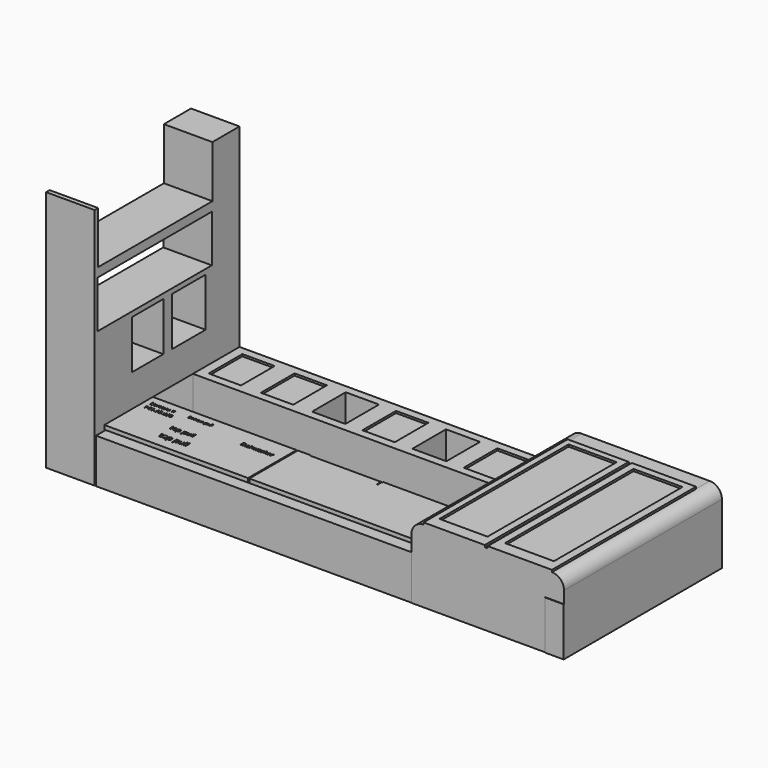
from build123d import *

# Parameters (mm, degrees)
F0_W      = 30
F0_H      = 720
F0_W_2    = 600
F0_W_3    = 400
F0_H_2    = 520
F0_W_4    = 411.4359617233
F0_W_5    = 420.5965995789
F0_W_6    = 110
F0_W_7    = 158.7504673004
F0_H_3    = 2090
F0_W_8    = 681.2495326996
F0_W_9    = 116.326417923
F0_W_10   = 783.673582077
F0_H_4    = 150
F1_DEPTH  = 600
F0_H_5    = 750
F0_W_11   = 5.8790212959
F0_H_6    = 38.7970095152
F0_W_12   = 5.4911354091
F0_H_7    = 47.2485832094
F0_W_13   = 564
F0_H_8    = 260
F0_W_14   = 7.9738955537
F0_H_9    = 74.7149404197
F0_W_15   = 6.7471420043
F0_H_10   = 63.2203305722
F0_W_16   = 4.4249870116
F0_H_11   = 41.461872519
F0_W_17   = 16
F0_W_18   = 1017
F0_W_19   = 1027
F0_W_20   = 878.7996225357
F0_H_12   = 70
F0_W_21   = 11.2003774643
F2_W      = 1887.2389125824
F2_H      = 600
F3_DEPTH  = 2440
F4_W      = 756.9127368927
F4_H      = 2226.2539291382
F4_W_2    = 594.5539474487
F4_H_2    = 1995.2517747879
F4_W_3    = 793.6194562912
F4_H_3    = 2227.2407436371
F4_W_4    = 605.0448417664
F4_H_4    = 1987.1687889099
F5_DEPTH  = 25
F6_START  = -200
F6_DEPTH  = 2080
F7_DEPTH  = 25
F8_DEPTH  = 25
F9_START  = -50
F9_DEPTH  = 550
F10_W     = 524.6109628677
F10_H     = 600
F10_W_2   = 133.528649807
F10_W_3   = 580.1107823849
F10_W_4   = 1763.4517922997
F10_H_2   = 584.0739011765
F10_W_5   = 720
F11_DEPTH = 600


with BuildPart() as f1:
    # F0 (on Top) → F1 (new body)
    with BuildSketch(Plane.XY):
        with Locations((27.8470897675, 1730)):
            Rectangle(F0_W, F0_H)
        with Locations((342.8470897675, 1730)):
            Rectangle(F0_W_2, F0_H)
        with Locations((327.3391544819, 1730)):
            Rectangle(F0_W_3, F0_H_2, mode=Mode.SUBTRACT)
        with Locations((657.8470897675, 1730)):
            Rectangle(F0_W, F0_H)
        with Locations((972.8470897675, 1730)):
            Rectangle(F0_W_2, F0_H)
        with Locations((972.8470897675, 1730)):
            Rectangle(F0_W_3, F0_H_2, mode=Mode.SUBTRACT)
        with Locations((1602.8470897675, 1730)):
            Rectangle(F0_W_2, F0_H)
        with Locations((1611.446917057, 1730)):
            Rectangle(F0_W_4, F0_H_2, mode=Mode.SUBTRACT)
        with Locations((2862.8470897675, 1730)):
            Rectangle(F0_W_2, F0_H)
        with Locations((2856.2989234924, 1730)):
            Rectangle(F0_W_5, F0_H_2, mode=Mode.SUBTRACT)
        with Locations((2547.8470897675, 1730)):
            Rectangle(F0_W, F0_H)
        with Locations((3177.8470897675, 1730)):
            Rectangle(F0_W, F0_H)
        with Locations((3492.8470897675, 1730)):
            Rectangle(F0_W_2, F0_H)
        with Locations((3480.6599140167, 1730)):
            Rectangle(F0_W_3, F0_H_2, mode=Mode.SUBTRACT)
        with Locations((3480.6599140167, 1730)):
            Rectangle(F0_W_3, F0_H_2)
        with Locations((3847.8470897675, 1730)):
            Rectangle(F0_W_6, F0_H)
        Polygon((3902.8470897675, 0), (3932.8470897675, 0), (3932.8470897675, 2090), (3902.8470897675, 2090), (3902.8470897675, 1370), align=None)
        with Locations((4012.2223234177, 1045)):
            Rectangle(F0_W_7, F0_H_3)
        Polygon((3932.8470897675, 2286.8287563324), (3932.8470897675, 2090), (4091.5975570679, 2090), (4772.8470897675, 2090), (4802.8470897675, 2090), (5586.5206718445, 2090), (5702.8470897675, 2090), (5820.0860023499, 2090), (5820.0860023499, 2286.8287563324), align=None)
        with Locations((4432.2223234177, 1045)):
            Rectangle(F0_W_8, F0_H_3)
        with Locations((4787.8470897675, 1045)):
            Rectangle(F0_W, F0_H_3)
        with Locations((5644.683880806, 1045)):
            Rectangle(F0_W_9, F0_H_3)
        with Locations((5194.683880806, 1045)):
            Rectangle(F0_W_10, F0_H_3)
        Polygon((5586.5206718445, 0), (5586.5206718445, -159.0223050117), (5820.0860023499, -159.0223050117), (5820.0860023499, 2090), (5702.8470897675, 2090), (5702.8470897675, 0), align=None)
        with Locations((327.3391544819, 1730)):
            Rectangle(F0_W_3, F0_H_2)
        with Locations((972.8470897675, 1730)):
            Rectangle(F0_W_3, F0_H_2)
        with Locations((2232.8470897675, 1730)):
            Rectangle(F0_W_2, F0_H)
        with Locations((2228.0454158783, 1730)):
            Rectangle(F0_W_3, F0_H_2, mode=Mode.SUBTRACT)
        with Locations((2228.0454158783, 1730)):
            Rectangle(F0_W_3, F0_H_2)
        with Locations((4012.2223234177, -75)):
            Rectangle(F0_W_7, F0_H_4)
        with Locations((1287.8470897675, 1730)):
            Rectangle(F0_W, F0_H)
        with Locations((1917.8470897675, 1730)):
            Rectangle(F0_W, F0_H)
    extrude(amount=-F1_DEPTH)

    # F2 (on face) → F3 (join)
    with BuildSketch(Plane(origin=(0, 2286.8287563324, 0), x_dir=(-1, 0, 0), z_dir=(0, 1, 0))):
        with BuildLine():
            Line((-5820.0860023499, 0), (-3932.8470897675, 0))
            Line((-3932.8470897675, 0), (-3932.8470897675, 150))
            ThreePointArc((-3932.8470897675, 150), (-3976.7810725895, 256.066017178), (-4082.8470897675, 300))
            Line((-4082.8470897675, 300), (-5670.0860023499, 300))
            ThreePointArc((-5670.0860023499, 300), (-5776.1520195278, 256.066017178), (-5820.0860023499, 150))
            Line((-5820.0860023499, 150), (-5820.0860023499, 0))
        make_face()
        with Locations((-4876.4665460587, -300)):
            Rectangle(F2_W, F2_H)
    extrude(amount=-F3_DEPTH)

    # F4 (on face) → F5 (join)
    with BuildSketch(Plane.XY.offset(300)):
        with Locations((4461.3034582138, 959.9557209015)):
            Rectangle(F4_W, F4_H)
        with Locations((4454.4014930725, 997.625887394)):
            Rectangle(F4_W_2, F4_H_2, mode=Mode.SUBTRACT)
        with Locations((5273.2762742043, 960.4491281509)):
            Rectangle(F4_W_3, F4_H_3)
        with Locations((5269.6921825409, 993.584394455)):
            Rectangle(F4_W_4, F4_H_4, mode=Mode.SUBTRACT)
    extrude(amount=F5_DEPTH)

    # F2 (on face) → F6 (join)
    with BuildSketch(Plane(origin=(0, 2286.8287563324, 0), x_dir=(-1, 0, 0), z_dir=(0, 1, 0)).offset(F6_START)):
        with BuildLine():
            Line((-3932.8470897675, 0), (-3932.8470897675, -600))
            Line((-3932.8470897675, -600), (-3803.3337593079, -600))
            Line((-3803.3337593079, -600), (-3803.3337593079, 1.4055977799))
            ThreePointArc((-3803.3337593079, 1.4055977799), (-3895.9244978361, 51.442911039), (-3932.8470897675, 150))
            Line((-3932.8470897675, 150), (-3932.8470897675, 0))
        make_face()
    extrude(amount=-F6_DEPTH)

    # F0 (on Top) → F7 (join)
    with BuildSketch(Plane.XY):
        with Locations((327.3391544819, 1730)):
            Rectangle(F0_W_3, F0_H_2)
        with Locations((972.8470897675, 1730)):
            Rectangle(F0_W_3, F0_H_2)
        with Locations((2228.0454158783, 1730)):
            Rectangle(F0_W_3, F0_H_2)
        with Locations((3480.6599140167, 1730)):
            Rectangle(F0_W_3, F0_H_2)
    extrude(amount=-F7_DEPTH)

    # F0 (on Top) → F8 (cut)
    with BuildSketch(Plane.XY):
        with Locations((327.3391544819, 1730)):
            Rectangle(F0_W_3, F0_H_2)
        with Locations((972.8470897675, 1730)):
            Rectangle(F0_W_3, F0_H_2)
        with Locations((2228.0454158783, 1730)):
            Rectangle(F0_W_3, F0_H_2)
        with Locations((3480.6599140167, 1730)):
            Rectangle(F0_W_3, F0_H_2)
    extrude(amount=-F8_DEPTH, mode=Mode.SUBTRACT)


with BuildPart() as f1b:
    # F0 (on Top) → F1, piece 2 (new body)
    with BuildSketch(Plane.XY):
        with Locations((1490, 375)):
            Rectangle(F0_W_2, F0_H_5)
        with BuildLine():
            add(Edge.make_bspline(
                [(1331.7365201631, 542.869279565), (1338.4254644314, 536.1803352968), (1338.4254644314, 524.1730856366)],
                knots=[0, 0, 0, 1, 1, 1], degree=2))
            add(Edge.make_bspline(
                [(1338.4254644314, 524.1730856366), (1338.4254644314, 511.3615768011), (1331.4703217037, 504.5820117807)],
                knots=[0, 0, 0, 1, 1, 1], degree=2))
            add(Edge.make_bspline(
                [(1331.4703217037, 504.5820117807), (1324.515178976, 497.8024467603), (1311.454463072, 497.8024467603)],
                knots=[0, 0, 0, 1, 1, 1], degree=2))
            Line((1311.454463072, 497.8024467603), (1297.1137290439, 497.8024467603))
            Line((1297.1137290439, 497.8024467603), (1297.1137290439, 549.5582238333))
            Line((1297.1137290439, 549.5582238333), (1312.9723606706, 549.5582238333))
            add(Edge.make_bspline(
                [(1312.9723606706, 549.5582238333), (1325.0475758949, 549.5582238333), (1331.7365201631, 542.869279565)],
                knots=[0, 0, 0, 1, 1, 1], degree=2))
        make_face(mode=Mode.SUBTRACT)
        with Locations((1352.0242410512, 517.2009515179)):
            Rectangle(F0_W_11, F0_H_6, mode=Mode.SUBTRACT)
        with BuildLine():
            add(Edge.make_bspline(
                [(1390.022655188, 514.7938377889), (1392.4467603081, 512.2451291346), (1392.4467603081, 508.3824195741)],
                knots=[0, 0, 0, 1, 1, 1], degree=2))
            add(Edge.make_bspline(
                [(1392.4467603081, 508.3824195741), (1392.4467603081, 502.967829633), (1388.4141368373, 500.028318985)],
                knots=[0, 0, 0, 1, 1, 1], degree=2))
            add(Edge.make_bspline(
                [(1388.4141368373, 500.028318985), (1384.3815133666, 497.0888083371), (1377.0865428183, 497.0888083371)],
                knots=[0, 0, 0, 1, 1, 1], degree=2))
            add(Edge.make_bspline(
                [(1377.0865428183, 497.0888083371), (1369.3724512913, 497.0888083371), (1365.0566379701, 499.5355686452)],
                knots=[0, 0, 0, 1, 1, 1], degree=2))
            Line((1365.0566379701, 499.5355686452), (1365.0566379701, 504.9841413684))
            add(Edge.make_bspline(
                [(1365.0566379701, 504.9841413684), (1367.8545536928, 503.568192116), (1371.0545990032, 502.7582691436)],
                knots=[0, 0, 0, 1, 1, 1], degree=2))
            add(Edge.make_bspline(
                [(1371.0545990032, 502.7582691436), (1374.2546443135, 501.9483461713), (1377.2338015406, 501.9483461713)],
                knots=[0, 0, 0, 1, 1, 1], degree=2))
            add(Edge.make_bspline(
                [(1377.2338015406, 501.9483461713), (1381.8328047123, 501.9483461713), (1384.3078840054, 503.4152695967)],
                knots=[0, 0, 0, 1, 1, 1], degree=2))
            add(Edge.make_bspline(
                [(1384.3078840054, 503.4152695967), (1386.7829632986, 504.8821930222), (1386.7829632986, 507.8953330313)],
                knots=[0, 0, 0, 1, 1, 1], degree=2))
            add(Edge.make_bspline(
                [(1386.7829632986, 507.8953330313), (1386.7829632986, 510.1608518351), (1384.8232895333, 511.7693701858)],
                knots=[0, 0, 0, 1, 1, 1], degree=2))
            add(Edge.make_bspline(
                [(1384.8232895333, 511.7693701858), (1382.863615768, 513.3778885365), (1377.1545083824, 515.5754417762)],
                knots=[0, 0, 0, 1, 1, 1], degree=2))
            add(Edge.make_bspline(
                [(1377.1545083824, 515.5754417762), (1371.7399184413, 517.5917535116), (1369.4574082465, 519.0983235161)],
                knots=[0, 0, 0, 1, 1, 1], degree=2))
            add(Edge.make_bspline(
                [(1369.4574082465, 519.0983235161), (1367.1748980517, 520.6048935206), (1366.0591300408, 522.5135931128)],
                knots=[0, 0, 0, 1, 1, 1], degree=2))
            add(Edge.make_bspline(
                [(1366.0591300408, 522.5135931128), (1364.9433620299, 524.422292705), (1364.9433620299, 527.0729497055)],
                knots=[0, 0, 0, 1, 1, 1], degree=2))
            add(Edge.make_bspline(
                [(1364.9433620299, 527.0729497055), (1364.9433620299, 531.8192115995), (1368.8060715904, 534.5661531491)],
                knots=[0, 0, 0, 1, 1, 1], degree=2))
            add(Edge.make_bspline(
                [(1368.8060715904, 534.5661531491), (1372.6687811509, 537.3130946987), (1379.3860444042, 537.3130946987)],
                knots=[0, 0, 0, 1, 1, 1], degree=2))
            add(Edge.make_bspline(
                [(1379.3860444042, 537.3130946987), (1385.6502038967, 537.3130946987), (1391.6425011328, 534.7643860444)],
                knots=[0, 0, 0, 1, 1, 1], degree=2))
            Line((1391.6425011328, 534.7643860444), (1389.5468962392, 529.9841413684))
            add(Edge.make_bspline(
                [(1389.5468962392, 529.9841413684), (1383.7131853194, 532.3855913004), (1378.9669234255, 532.3855913004)],
                knots=[0, 0, 0, 1, 1, 1], degree=2))
            add(Edge.make_bspline(
                [(1378.9669234255, 532.3855913004), (1374.7870412324, 532.3855913004), (1372.6631173539, 531.0772541912)],
                knots=[0, 0, 0, 1, 1, 1], degree=2))
            add(Edge.make_bspline(
                [(1372.6631173539, 531.0772541912), (1370.5391934753, 529.768917082), (1370.5391934753, 527.4694154961)],
                knots=[0, 0, 0, 1, 1, 1], degree=2))
            add(Edge.make_bspline(
                [(1370.5391934753, 527.4694154961), (1370.5391934753, 525.9062075215), (1371.3377888536, 524.8130946987)],
                knots=[0, 0, 0, 1, 1, 1], degree=2))
            add(Edge.make_bspline(
                [(1371.3377888536, 524.8130946987), (1372.136384232, 523.7199818758), (1373.903488899, 522.7288173992)],
                knots=[0, 0, 0, 1, 1, 1], degree=2))
            add(Edge.make_bspline(
                [(1373.903488899, 522.7288173992), (1375.6705935659, 521.7376529225), (1380.7000453104, 519.8572723154)],
                knots=[0, 0, 0, 1, 1, 1], degree=2))
            add(Edge.make_bspline(
                [(1380.7000453104, 519.8572723154), (1387.598550068, 517.3425464431), (1390.022655188, 514.7938377889)],
                knots=[0, 0, 0, 1, 1, 1], degree=2))
        make_face(mode=Mode.SUBTRACT)
        with BuildLine():
            Line((1434.4381513367, 497.8024467603), (1428.5591300408, 497.8024467603))
            Line((1428.5591300408, 497.8024467603), (1428.5591300408, 522.9043951065))
            add(Edge.make_bspline(
                [(1428.5591300408, 522.9043951065), (1428.5591300408, 527.6393294064), (1426.4012233802, 529.9784775714)],
                knots=[0, 0, 0, 1, 1, 1], degree=2))
            add(Edge.make_bspline(
                [(1426.4012233802, 529.9784775714), (1424.2433167195, 532.3176257363), (1419.6329859538, 532.3176257363)],
                knots=[0, 0, 0, 1, 1, 1], degree=2))
            add(Edge.make_bspline(
                [(1419.6329859538, 532.3176257363), (1413.5160851835, 532.3176257363), (1410.7011780698, 528.9873130947)],
                knots=[0, 0, 0, 1, 1, 1], degree=2))
            add(Edge.make_bspline(
                [(1410.7011780698, 528.9873130947), (1407.886270956, 525.6570004531), (1407.886270956, 518.0901676484)],
                knots=[0, 0, 0, 1, 1, 1], degree=2))
            Line((1407.886270956, 518.0901676484), (1407.886270956, 497.8024467603))
            Line((1407.886270956, 497.8024467603), (1402.0072496602, 497.8024467603))
            Line((1402.0072496602, 497.8024467603), (1402.0072496602, 552.8885364749))
            Line((1402.0072496602, 552.8885364749), (1407.886270956, 552.8885364749))
            Line((1407.886270956, 552.8885364749), (1407.886270956, 536.2143180788))
            add(Edge.make_bspline(
                [(1407.886270956, 536.2143180788), (1407.886270956, 533.2011780698), (1407.6030811056, 531.2188491164)],
                knots=[0, 0, 0, 1, 1, 1], degree=2))
            Line((1407.6030811056, 531.2188491164), (1407.9542365202, 531.2188491164))
            add(Edge.make_bspline(
                [(1407.9542365202, 531.2188491164), (1409.6873584051, 534.0167648391), (1412.8930675125, 535.6252831899)],
                knots=[0, 0, 0, 1, 1, 1], degree=2))
            add(Edge.make_bspline(
                [(1412.8930675125, 535.6252831899), (1416.0987766198, 537.2338015406), (1420.1993656547, 537.2338015406)],
                knots=[0, 0, 0, 1, 1, 1], degree=2))
            add(Edge.make_bspline(
                [(1420.1993656547, 537.2338015406), (1427.3130946987, 537.2338015406), (1430.8756230177, 533.8525147259)],
                knots=[0, 0, 0, 1, 1, 1], degree=2))
            add(Edge.make_bspline(
                [(1430.8756230177, 533.8525147259), (1434.4381513367, 530.4712279112), (1434.4381513367, 523.1082917988)],
                knots=[0, 0, 0, 1, 1, 1], degree=2))
            Line((1434.4381513367, 523.1082917988), (1434.4381513367, 497.8024467603))
        make_face(mode=Mode.SUBTRACT)
        with BuildLine():
            add(Edge.make_bspline(
                [(1349.5774807431, 544.1549614862), (1348.5863162664, 545.1291345718), (1348.5863162664, 547.1114635251)],
                knots=[0, 0, 0, 1, 1, 1], degree=2))
            add(Edge.make_bspline(
                [(1348.5863162664, 547.1114635251), (1348.5863162664, 549.1277752605), (1349.5774807431, 550.0679655641)],
                knots=[0, 0, 0, 1, 1, 1], degree=2))
            add(Edge.make_bspline(
                [(1349.5774807431, 550.0679655641), (1350.5686452198, 551.0081558677), (1352.0638876303, 551.0081558677)],
                knots=[0, 0, 0, 1, 1, 1], degree=2))
            add(Edge.make_bspline(
                [(1352.0638876303, 551.0081558677), (1353.4798368826, 551.0081558677), (1354.5049841414, 550.0509741731)],
                knots=[0, 0, 0, 1, 1, 1], degree=2))
            add(Edge.make_bspline(
                [(1354.5049841414, 550.0509741731), (1355.5301314001, 549.0937924785), (1355.5301314001, 547.1114635251)],
                knots=[0, 0, 0, 1, 1, 1], degree=2))
            add(Edge.make_bspline(
                [(1355.5301314001, 547.1114635251), (1355.5301314001, 545.1291345718), (1354.5049841414, 544.1549614862)],
                knots=[0, 0, 0, 1, 1, 1], degree=2))
            add(Edge.make_bspline(
                [(1354.5049841414, 544.1549614862), (1353.4798368826, 543.1807884005), (1352.0638876303, 543.1807884005)],
                knots=[0, 0, 0, 1, 1, 1], degree=2))
            add(Edge.make_bspline(
                [(1352.0638876303, 543.1807884005), (1350.5686452198, 543.1807884005), (1349.5774807431, 544.1549614862)],
                knots=[0, 0, 0, 1, 1, 1], degree=2))
        make_face(mode=Mode.SUBTRACT)
        with BuildLine():
            Line((1485.1631173539, 497.8024467603), (1478.1853194381, 497.8024467603))
            Line((1478.1853194381, 497.8024467603), (1471.0715903942, 520.5595831445))
            add(Edge.make_bspline(
                [(1471.0715903942, 520.5595831445), (1470.3919347531, 522.6551880381), (1468.556864522, 530.0521069325)],
                knots=[0, 0, 0, 1, 1, 1], degree=2))
            Line((1468.556864522, 530.0521069325), (1468.2736746715, 530.0521069325))
            add(Edge.make_bspline(
                [(1468.2736746715, 530.0521069325), (1466.8577254191, 523.8559130041), (1465.7929315813, 520.4916175804)],
                knots=[0, 0, 0, 1, 1, 1], degree=2))
            Line((1465.7929315813, 520.4916175804), (1458.463978251, 497.8024467603))
            Line((1458.463978251, 497.8024467603), (1451.6674218396, 497.8024467603))
            Line((1451.6674218396, 497.8024467603), (1441.0874490258, 536.5994562755))
            Line((1441.0874490258, 536.5994562755), (1447.2496601722, 536.5994562755))
            add(Edge.make_bspline(
                [(1447.2496601722, 536.5994562755), (1450.9990937925, 521.9755323969), (1452.9644313548, 514.3294064341)],
                knots=[0, 0, 0, 1, 1, 1], degree=2))
            add(Edge.make_bspline(
                [(1452.9644313548, 514.3294064341), (1454.9297689171, 506.6832804712), (1455.2129587676, 504.0326234708)],
                knots=[0, 0, 0, 1, 1, 1], degree=2))
            Line((1455.2129587676, 504.0326234708), (1455.496148618, 504.0326234708))
            add(Edge.make_bspline(
                [(1455.496148618, 504.0326234708), (1455.8812868147, 506.0489352062), (1456.7478477571, 509.2546443135)],
                knots=[0, 0, 0, 1, 1, 1], degree=2))
            add(Edge.make_bspline(
                [(1456.7478477571, 509.2546443135), (1457.6144086996, 512.4603534209), (1458.2600815587, 514.3294064341)],
                knots=[0, 0, 0, 1, 1, 1], degree=2))
            Line((1458.2600815587, 514.3294064341), (1465.3738106026, 536.5994562755))
            Line((1465.3738106026, 536.5994562755), (1471.7399184413, 536.5994562755))
            Line((1471.7399184413, 536.5994562755), (1478.683733575, 514.3294064341))
            add(Edge.make_bspline(
                [(1478.683733575, 514.3294064341), (1480.6660625283, 508.2464884459), (1481.3683733575, 504.1005890349)],
                knots=[0, 0, 0, 1, 1, 1], degree=2))
            Line((1481.3683733575, 504.1005890349), (1481.651563208, 504.1005890349))
            add(Edge.make_bspline(
                [(1481.651563208, 504.1005890349), (1481.7988219302, 505.380607159), (1482.4161758043, 508.0369279565)],
                knots=[0, 0, 0, 1, 1, 1], degree=2))
            add(Edge.make_bspline(
                [(1482.4161758043, 508.0369279565), (1483.0335296783, 510.693248754), (1489.7961033077, 536.5994562755)],
                knots=[0, 0, 0, 1, 1, 1], degree=2))
            Line((1489.7961033077, 536.5994562755), (1495.8790212959, 536.5994562755))
            Line((1495.8790212959, 536.5994562755), (1485.1631173539, 497.8024467603))
        make_face(mode=Mode.SUBTRACT)
        with BuildLine():
            Line((1531.1078386951, 497.8024467603), (1526.7467149977, 497.8024467603))
            Line((1526.7467149977, 497.8024467603), (1525.5799728138, 503.3303126416))
            Line((1525.5799728138, 503.3303126416), (1525.2967829633, 503.3303126416))
            add(Edge.make_bspline(
                [(1525.2967829633, 503.3303126416), (1522.3969188944, 499.6828273675), (1519.5140462166, 498.3858178523)],
                knots=[0, 0, 0, 1, 1, 1], degree=2))
            add(Edge.make_bspline(
                [(1519.5140462166, 498.3858178523), (1516.6311735387, 497.0888083371), (1512.3040326235, 497.0888083371)],
                knots=[0, 0, 0, 1, 1, 1], degree=2))
            add(Edge.make_bspline(
                [(1512.3040326235, 497.0888083371), (1506.5382872678, 497.0888083371), (1503.2646125963, 500.0679655641)],
                knots=[0, 0, 0, 1, 1, 1], degree=2))
            add(Edge.make_bspline(
                [(1503.2646125963, 500.0679655641), (1499.9909379248, 503.0471227911), (1499.9909379248, 508.5296782963)],
                knots=[0, 0, 0, 1, 1, 1], degree=2))
            add(Edge.make_bspline(
                [(1499.9909379248, 508.5296782963), (1499.9909379248, 520.2763932941), (1518.7834164024, 520.842772995)],
                knots=[0, 0, 0, 1, 1, 1], degree=2))
            Line((1518.7834164024, 520.842772995), (1525.3647485274, 521.0579972814))
            Line((1525.3647485274, 521.0579972814), (1525.3647485274, 523.4707748074))
            add(Edge.make_bspline(
                [(1525.3647485274, 523.4707748074), (1525.3647485274, 528.0357951971), (1523.4050747621, 530.2106932488)],
                knots=[0, 0, 0, 1, 1, 1], degree=2))
            add(Edge.make_bspline(
                [(1523.4050747621, 530.2106932488), (1521.4454009968, 532.3855913004), (1517.1182600816, 532.3855913004)],
                knots=[0, 0, 0, 1, 1, 1], degree=2))
            add(Edge.make_bspline(
                [(1517.1182600816, 532.3855913004), (1512.2700498414, 532.3855913004), (1506.1531490711, 529.4177616674)],
                knots=[0, 0, 0, 1, 1, 1], degree=2))
            Line((1506.1531490711, 529.4177616674), (1504.3407340281, 533.914816493))
            add(Edge.make_bspline(
                [(1504.3407340281, 533.914816493), (1507.2066153149, 535.4666968736), (1510.6218849116, 536.3502492071)],
                knots=[0, 0, 0, 1, 1, 1], degree=2))
            add(Edge.make_bspline(
                [(1510.6218849116, 536.3502492071), (1514.0371545084, 537.2338015406), (1517.4807430902, 537.2338015406)],
                knots=[0, 0, 0, 1, 1, 1], degree=2))
            add(Edge.make_bspline(
                [(1517.4807430902, 537.2338015406), (1524.4132306298, 537.2338015406), (1527.7605346624, 534.1583597644)],
                knots=[0, 0, 0, 1, 1, 1], degree=2))
            add(Edge.make_bspline(
                [(1527.7605346624, 534.1583597644), (1531.1078386951, 531.0829179882), (1531.1078386951, 524.2863615768)],
                knots=[0, 0, 0, 1, 1, 1], degree=2))
            Line((1531.1078386951, 524.2863615768), (1531.1078386951, 497.8024467603))
        make_face(mode=Mode.SUBTRACT)
        with BuildLine():
            add(Edge.make_bspline(
                [(1565.8042591753, 514.7938377889), (1568.2283642954, 512.2451291346), (1568.2283642954, 508.3824195741)],
                knots=[0, 0, 0, 1, 1, 1], degree=2))
            add(Edge.make_bspline(
                [(1568.2283642954, 508.3824195741), (1568.2283642954, 502.967829633), (1564.1957408246, 500.028318985)],
                knots=[0, 0, 0, 1, 1, 1], degree=2))
            add(Edge.make_bspline(
                [(1564.1957408246, 500.028318985), (1560.1631173539, 497.0888083371), (1552.8681468056, 497.0888083371)],
                knots=[0, 0, 0, 1, 1, 1], degree=2))
            add(Edge.make_bspline(
                [(1552.8681468056, 497.0888083371), (1545.1540552787, 497.0888083371), (1540.8382419574, 499.5355686452)],
                knots=[0, 0, 0, 1, 1, 1], degree=2))
            Line((1540.8382419574, 499.5355686452), (1540.8382419574, 504.9841413684))
            add(Edge.make_bspline(
                [(1540.8382419574, 504.9841413684), (1543.6361576801, 503.568192116), (1546.8362029905, 502.7582691436)],
                knots=[0, 0, 0, 1, 1, 1], degree=2))
            add(Edge.make_bspline(
                [(1546.8362029905, 502.7582691436), (1550.0362483009, 501.9483461713), (1553.0154055279, 501.9483461713)],
                knots=[0, 0, 0, 1, 1, 1], degree=2))
            add(Edge.make_bspline(
                [(1553.0154055279, 501.9483461713), (1557.6144086996, 501.9483461713), (1560.0894879927, 503.4152695967)],
                knots=[0, 0, 0, 1, 1, 1], degree=2))
            add(Edge.make_bspline(
                [(1560.0894879927, 503.4152695967), (1562.5645672859, 504.8821930222), (1562.5645672859, 507.8953330313)],
                knots=[0, 0, 0, 1, 1, 1], degree=2))
            add(Edge.make_bspline(
                [(1562.5645672859, 507.8953330313), (1562.5645672859, 510.1608518351), (1560.6048935206, 511.7693701858)],
                knots=[0, 0, 0, 1, 1, 1], degree=2))
            add(Edge.make_bspline(
                [(1560.6048935206, 511.7693701858), (1558.6452197553, 513.3778885365), (1552.9361123697, 515.5754417762)],
                knots=[0, 0, 0, 1, 1, 1], degree=2))
            add(Edge.make_bspline(
                [(1552.9361123697, 515.5754417762), (1547.5215224286, 517.5917535116), (1545.2390122338, 519.0983235161)],
                knots=[0, 0, 0, 1, 1, 1], degree=2))
            add(Edge.make_bspline(
                [(1545.2390122338, 519.0983235161), (1542.956502039, 520.6048935206), (1541.8407340281, 522.5135931128)],
                knots=[0, 0, 0, 1, 1, 1], degree=2))
            add(Edge.make_bspline(
                [(1541.8407340281, 522.5135931128), (1540.7249660172, 524.422292705), (1540.7249660172, 527.0729497055)],
                knots=[0, 0, 0, 1, 1, 1], degree=2))
            add(Edge.make_bspline(
                [(1540.7249660172, 527.0729497055), (1540.7249660172, 531.8192115995), (1544.5876755777, 534.5661531491)],
                knots=[0, 0, 0, 1, 1, 1], degree=2))
            add(Edge.make_bspline(
                [(1544.5876755777, 534.5661531491), (1548.4503851382, 537.3130946987), (1555.1676483915, 537.3130946987)],
                knots=[0, 0, 0, 1, 1, 1], degree=2))
            add(Edge.make_bspline(
                [(1555.1676483915, 537.3130946987), (1561.431807884, 537.3130946987), (1567.4241051201, 534.7643860444)],
                knots=[0, 0, 0, 1, 1, 1], degree=2))
            Line((1567.4241051201, 534.7643860444), (1565.3285002266, 529.9841413684))
            add(Edge.make_bspline(
                [(1565.3285002266, 529.9841413684), (1559.4947893067, 532.3855913004), (1554.7485274128, 532.3855913004)],
                knots=[0, 0, 0, 1, 1, 1], degree=2))
            add(Edge.make_bspline(
                [(1554.7485274128, 532.3855913004), (1550.5686452198, 532.3855913004), (1548.4447213412, 531.0772541912)],
                knots=[0, 0, 0, 1, 1, 1], degree=2))
            add(Edge.make_bspline(
                [(1548.4447213412, 531.0772541912), (1546.3207974626, 529.768917082), (1546.3207974626, 527.4694154961)],
                knots=[0, 0, 0, 1, 1, 1], degree=2))
            add(Edge.make_bspline(
                [(1546.3207974626, 527.4694154961), (1546.3207974626, 525.9062075215), (1547.119392841, 524.8130946987)],
                knots=[0, 0, 0, 1, 1, 1], degree=2))
            add(Edge.make_bspline(
                [(1547.119392841, 524.8130946987), (1547.9179882193, 523.7199818758), (1549.6850928863, 522.7288173992)],
                knots=[0, 0, 0, 1, 1, 1], degree=2))
            add(Edge.make_bspline(
                [(1549.6850928863, 522.7288173992), (1551.4521975532, 521.7376529225), (1556.4816492977, 519.8572723154)],
                knots=[0, 0, 0, 1, 1, 1], degree=2))
            add(Edge.make_bspline(
                [(1556.4816492977, 519.8572723154), (1563.3801540553, 517.3425464431), (1565.8042591753, 514.7938377889)],
                knots=[0, 0, 0, 1, 1, 1], degree=2))
        make_face(mode=Mode.SUBTRACT)
        with BuildLine():
            add(Edge.make_bspline(
                [(1645.380607159, 497.6778432261), (1642.6053466244, 497.0888083371), (1638.6746714998, 497.0888083371)],
                knots=[0, 0, 0, 1, 1, 1], degree=2))
            add(Edge.make_bspline(
                [(1638.6746714998, 497.0888083371), (1630.0770276393, 497.0888083371), (1625.098550068, 502.3334843679)],
                knots=[0, 0, 0, 1, 1, 1], degree=2))
            add(Edge.make_bspline(
                [(1625.098550068, 502.3334843679), (1620.1200724966, 507.5781603987), (1620.1200724966, 516.8781150884)],
                knots=[0, 0, 0, 1, 1, 1], degree=2))
            add(Edge.make_bspline(
                [(1620.1200724966, 516.8781150884), (1620.1200724966, 526.2686905301), (1624.7417308564, 531.7908926144)],
                knots=[0, 0, 0, 1, 1, 1], degree=2))
            add(Edge.make_bspline(
                [(1624.7417308564, 531.7908926144), (1629.3633892161, 537.3130946987), (1637.1567739012, 537.3130946987)],
                knots=[0, 0, 0, 1, 1, 1], degree=2))
            add(Edge.make_bspline(
                [(1637.1567739012, 537.3130946987), (1644.4404168555, 537.3130946987), (1648.6882646126, 532.5158586316)],
                knots=[0, 0, 0, 1, 1, 1], degree=2))
            add(Edge.make_bspline(
                [(1648.6882646126, 532.5158586316), (1652.9361123697, 527.7186225646), (1652.9361123697, 519.8572723154)],
                knots=[0, 0, 0, 1, 1, 1], degree=2))
            Line((1652.9361123697, 519.8572723154), (1652.9361123697, 516.1418214771))
            Line((1652.9361123697, 516.1418214771), (1626.2143180788, 516.1418214771))
            add(Edge.make_bspline(
                [(1626.2143180788, 516.1418214771), (1626.3955595831, 509.3112822836), (1629.6692342546, 505.7714091527)],
                knots=[0, 0, 0, 1, 1, 1], degree=2))
            add(Edge.make_bspline(
                [(1629.6692342546, 505.7714091527), (1632.9429089261, 502.2315360217), (1638.8898957861, 502.2315360217)],
                knots=[0, 0, 0, 1, 1, 1], degree=2))
            add(Edge.make_bspline(
                [(1638.8898957861, 502.2315360217), (1645.1540552787, 502.2315360217), (1651.2709560489, 504.8482102401)],
                knots=[0, 0, 0, 1, 1, 1], degree=2))
            Line((1651.2709560489, 504.8482102401), (1651.2709560489, 499.6035342093))
            add(Edge.make_bspline(
                [(1651.2709560489, 499.6035342093), (1648.1558676937, 498.2668781151), (1645.380607159, 497.6778432261)],
                knots=[0, 0, 0, 1, 1, 1], degree=2))
        make_face(mode=Mode.SUBTRACT)
        with BuildLine():
            Line((1610.219755324, 497.8024467603), (1604.3407340281, 497.8024467603))
            Line((1604.3407340281, 497.8024467603), (1604.3407340281, 522.9043951065))
            add(Edge.make_bspline(
                [(1604.3407340281, 522.9043951065), (1604.3407340281, 527.6393294064), (1602.1828273675, 529.9784775714)],
                knots=[0, 0, 0, 1, 1, 1], degree=2))
            add(Edge.make_bspline(
                [(1602.1828273675, 529.9784775714), (1600.0249207068, 532.3176257363), (1595.4145899411, 532.3176257363)],
                knots=[0, 0, 0, 1, 1, 1], degree=2))
            add(Edge.make_bspline(
                [(1595.4145899411, 532.3176257363), (1589.2976891708, 532.3176257363), (1586.4827820571, 528.9873130947)],
                knots=[0, 0, 0, 1, 1, 1], degree=2))
            add(Edge.make_bspline(
                [(1586.4827820571, 528.9873130947), (1583.6678749434, 525.6570004531), (1583.6678749434, 518.0901676484)],
                knots=[0, 0, 0, 1, 1, 1], degree=2))
            Line((1583.6678749434, 518.0901676484), (1583.6678749434, 497.8024467603))
            Line((1583.6678749434, 497.8024467603), (1577.7888536475, 497.8024467603))
            Line((1577.7888536475, 497.8024467603), (1577.7888536475, 552.8885364749))
            Line((1577.7888536475, 552.8885364749), (1583.6678749434, 552.8885364749))
            Line((1583.6678749434, 552.8885364749), (1583.6678749434, 536.2143180788))
            add(Edge.make_bspline(
                [(1583.6678749434, 536.2143180788), (1583.6678749434, 533.2011780698), (1583.3846850929, 531.2188491164)],
                knots=[0, 0, 0, 1, 1, 1], degree=2))
            Line((1583.3846850929, 531.2188491164), (1583.7358405075, 531.2188491164))
            add(Edge.make_bspline(
                [(1583.7358405075, 531.2188491164), (1585.4689623924, 534.0167648391), (1588.6746714998, 535.6252831899)],
                knots=[0, 0, 0, 1, 1, 1], degree=2))
            add(Edge.make_bspline(
                [(1588.6746714998, 535.6252831899), (1591.8803806072, 537.2338015406), (1595.980969642, 537.2338015406)],
                knots=[0, 0, 0, 1, 1, 1], degree=2))
            add(Edge.make_bspline(
                [(1595.980969642, 537.2338015406), (1603.094698686, 537.2338015406), (1606.657227005, 533.8525147259)],
                knots=[0, 0, 0, 1, 1, 1], degree=2))
            add(Edge.make_bspline(
                [(1606.657227005, 533.8525147259), (1610.219755324, 530.4712279112), (1610.219755324, 523.1082917988)],
                knots=[0, 0, 0, 1, 1, 1], degree=2))
            Line((1610.219755324, 523.1082917988), (1610.219755324, 497.8024467603))
        make_face(mode=Mode.SUBTRACT)
        with BuildLine():
            add(Edge.make_bspline(
                [(1673.9714544631, 535.2571363842), (1677.0185772542, 537.3130946987), (1680.6660625283, 537.3130946987)],
                knots=[0, 0, 0, 1, 1, 1], degree=2))
            add(Edge.make_bspline(
                [(1680.6660625283, 537.3130946987), (1683.2487539647, 537.3130946987), (1685.2990484821, 536.882646126)],
                knots=[0, 0, 0, 1, 1, 1], degree=2))
            Line((1685.2990484821, 536.882646126), (1684.4834617127, 531.4340734028))
            add(Edge.make_bspline(
                [(1684.4834617127, 531.4340734028), (1682.0820117807, 531.9664703217), (1680.2356139556, 531.9664703217)],
                knots=[0, 0, 0, 1, 1, 1], degree=2))
            add(Edge.make_bspline(
                [(1680.2356139556, 531.9664703217), (1675.5233348437, 531.9664703217), (1672.1816946081, 528.1434073403)],
                knots=[0, 0, 0, 1, 1, 1], degree=2))
            add(Edge.make_bspline(
                [(1672.1816946081, 528.1434073403), (1668.8400543724, 524.3203443589), (1668.8400543724, 518.6225645673)],
                knots=[0, 0, 0, 1, 1, 1], degree=2))
            Line((1668.8400543724, 518.6225645673), (1668.8400543724, 497.8024467603))
            Line((1668.8400543724, 497.8024467603), (1662.9610330766, 497.8024467603))
            Line((1662.9610330766, 497.8024467603), (1662.9610330766, 536.5994562755))
            Line((1662.9610330766, 536.5994562755), (1667.8092433167, 536.5994562755))
            Line((1667.8092433167, 536.5994562755), (1668.4888989579, 529.4177616674))
            Line((1668.4888989579, 529.4177616674), (1668.7720888083, 529.4177616674))
            add(Edge.make_bspline(
                [(1668.7720888083, 529.4177616674), (1670.924331672, 533.2011780698), (1673.9714544631, 535.2571363842)],
                knots=[0, 0, 0, 1, 1, 1], degree=2))
        make_face(mode=Mode.SUBTRACT)
        with BuildLine():
            Line((590, 750), (30, 750))
            Line((30, 750), (30, 0))
            Line((30, 0), (590, 0))
            Line((590, 0), (590, 144.479632282))
            add(Edge.make_bspline(
                [(590, 144.479632282), (589.4652171861, 144.3683430494), (588.8593756924, 144.2686008522)],
                knots=[0.7595570865, 0.7595570865, 0.7595570865, 1, 1, 1], degree=2))
            add(Edge.make_bspline(
                [(588.8593756924, 144.2686008522), (586.3396861532, 143.8537739159), (584.3116433534, 143.8537739159)],
                knots=[0, 0, 0, 1, 1, 1], degree=2))
            add(Edge.make_bspline(
                [(584.3116433534, 143.8537739159), (569.0552304732, 143.8537739159), (569.0552304732, 159.9398406688)],
                knots=[0, 0, 0, 1, 1, 1], degree=2))
            Line((569.0552304732, 159.9398406688), (569.0552304732, 191.2515923808))
            Line((569.0552304732, 191.2515923808), (561.5115258164, 191.2515923808))
            Line((561.5115258164, 191.2515923808), (561.5115258164, 195.0925825319))
            Line((561.5115258164, 195.0925825319), (569.0552304732, 198.4111980225))
            Line((569.0552304732, 198.4111980225), (572.4045738849, 209.6422532243))
            Line((572.4045738849, 209.6422532243), (577.0137620663, 209.6422532243))
            Line((577.0137620663, 209.6422532243), (577.0137620663, 197.4432685044))
            Line((577.0137620663, 197.4432685044), (590, 197.4432685044))
            Line((590, 197.4432685044), (590, 336.1018430902))
            add(Edge.make_bspline(
                [(590, 336.1018430902), (588.6454461734, 336.6568510427), (587.3903295724, 337.4183824635)],
                knots=[0.7288050594, 0.7288050594, 0.7288050594, 1, 1, 1], degree=2))
            add(Edge.make_bspline(
                [(587.3903295724, 337.4183824635), (582.7622321667, 340.2264415636), (580.2401790861, 345.465551829)],
                knots=[0, 0, 0, 1, 1, 1], degree=2))
            add(Edge.make_bspline(
                [(580.2401790861, 345.465551829), (577.7181260055, 350.7046620944), (577.7181260055, 357.7378101181)],
                knots=[0, 0, 0, 1, 1, 1], degree=2))
            add(Edge.make_bspline(
                [(577.7181260055, 357.7378101181), (577.7181260055, 368.6190391309), (583.1652406487, 374.6966670442)],
                knots=[0, 0, 0, 1, 1, 1], degree=2))
            add(Edge.make_bspline(
                [(583.1652406487, 374.6966670442), (586.0074608573, 377.8678793295), (590, 379.3844020711)],
                knots=[0, 0, 0, 0.52178454, 0.52178454, 0.52178454], degree=2))
            Line((590, 379.3844020711), (590, 621.0368930993))
            add(Edge.make_bspline(
                [(590, 621.0368930993), (587.676978186, 621.4590359557), (585.7218604069, 622.6452871924)],
                knots=[0.3558629431, 0.3558629431, 0.3558629431, 1, 1, 1], degree=2))
            add(Edge.make_bspline(
                [(585.7218604069, 622.6452871924), (582.6866092005, 624.486900284), (581.0325678128, 627.9228728575)],
                knots=[0, 0, 0, 1, 1, 1], degree=2))
            add(Edge.make_bspline(
                [(581.0325678128, 627.9228728575), (579.378526425, 631.358845431), (579.378526425, 635.9714041464)],
                knots=[0, 0, 0, 1, 1, 1], degree=2))
            add(Edge.make_bspline(
                [(579.378526425, 635.9714041464), (579.378526425, 643.1076548761), (582.9509147831, 647.0935535811)],
                knots=[0, 0, 0, 1, 1, 1], degree=2))
            add(Edge.make_bspline(
                [(582.9509147831, 647.0935535811), (585.6717648965, 650.1293469654), (590, 650.8529788639)],
                knots=[0, 0, 0, 0.7616333502, 0.7616333502, 0.7616333502], degree=2))
            Line((590, 650.8529788639), (590, 750))
        make_face()
        with BuildLine():
            add(Edge.make_bspline(
                [(559.9727525259, 342.3389860254), (561.8837927468, 340.1874407427), (565.2118627913, 340.1874407427)],
                knots=[0, 0, 0, 1, 1, 1], degree=2))
            add(Edge.make_bspline(
                [(565.2118627913, 340.1874407427), (567.0059005497, 340.1874407427), (568.669935572, 340.447446215)],
                knots=[0, 0, 0, 1, 1, 1], degree=2))
            add(Edge.make_bspline(
                [(568.669935572, 340.447446215), (570.3339705942, 340.7074516872), (571.3089911151, 340.9934577066)],
                knots=[0, 0, 0, 1, 1, 1], degree=2))
            Line((571.3089911151, 340.9934577066), (571.3089911151, 335.8323490829))
            add(Edge.make_bspline(
                [(571.3089911151, 335.8323490829), (570.2169681317, 335.3123381385), (568.0849232594, 334.961330751)],
                knots=[0, 0, 0, 1, 1, 1], degree=2))
            add(Edge.make_bspline(
                [(568.0849232594, 334.961330751), (565.9528783872, 334.6103233634), (564.2368422705, 334.6103233634)],
                knots=[0, 0, 0, 1, 1, 1], degree=2))
            add(Edge.make_bspline(
                [(564.2368422705, 334.6103233634), (551.3275705744, 334.6103233634), (551.3275705744, 348.2216098346)],
                knots=[0, 0, 0, 1, 1, 1], degree=2))
            Line((551.3275705744, 348.2216098346), (551.3275705744, 374.7161674546))
            Line((551.3275705744, 374.7161674546), (544.9444362312, 374.7161674546))
            Line((544.9444362312, 374.7161674546), (544.9444362312, 377.9662358575))
            Line((544.9444362312, 377.9662358575), (551.3275705744, 380.7742949575))
            Line((551.3275705744, 380.7742949575), (554.1616302216, 390.2774949674))
            Line((554.1616302216, 390.2774949674), (558.0617123051, 390.2774949674))
            Line((558.0617123051, 390.2774949674), (558.0617123051, 379.95527772))
            Line((558.0617123051, 379.95527772), (570.9839842748, 379.95527772))
            Line((570.9839842748, 379.95527772), (570.9839842748, 374.7161674546))
            Line((570.9839842748, 374.7161674546), (558.0617123051, 374.7161674546))
            Line((558.0617123051, 374.7161674546), (558.0617123051, 348.507615854))
            add(Edge.make_bspline(
                [(558.0617123051, 348.507615854), (558.0617123051, 344.4905313081), (559.9727525259, 342.3389860254)],
                knots=[0, 0, 0, 1, 1, 1], degree=2))
        make_face(mode=Mode.SUBTRACT)
        with BuildLine():
            add(Edge.make_bspline(
                [(199.5071682774, 523.0451088994), (198.4265211018, 524.0637093472), (198.4265211018, 526.3904616392)],
                knots=[0, 0, 0, 1, 1, 1], degree=2))
            add(Edge.make_bspline(
                [(198.4265211018, 526.3904616392), (198.4265211018, 528.5620971117), (199.4140981857, 529.6737676512)],
                knots=[0, 0, 0, 1, 1, 1], degree=2))
            add(Edge.make_bspline(
                [(199.4140981857, 529.6737676512), (200.4016752696, 530.7854381907), (202.2423948606, 530.7854381907)],
                knots=[0, 0, 0, 1, 1, 1], degree=2))
            add(Edge.make_bspline(
                [(202.2423948606, 530.7854381907), (204.1141378155, 530.7854381907), (205.1637616272, 529.6737676512)],
                knots=[0, 0, 0, 1, 1, 1], degree=2))
            add(Edge.make_bspline(
                [(205.1637616272, 529.6737676512), (206.213385439, 528.5620971117), (206.213385439, 526.3904616392)],
                knots=[0, 0, 0, 1, 1, 1], degree=2))
            add(Edge.make_bspline(
                [(206.213385439, 526.3904616392), (206.213385439, 524.2912140157), (205.1482499453, 523.1588612336)],
                knots=[0, 0, 0, 1, 1, 1], degree=2))
            add(Edge.make_bspline(
                [(205.1482499453, 523.1588612336), (204.0831144516, 522.0265084515), (202.2423948606, 522.0265084515)],
                knots=[0, 0, 0, 1, 1, 1], degree=2))
            add(Edge.make_bspline(
                [(202.2423948606, 522.0265084515), (200.587815453, 522.0265084515), (199.5071682774, 523.0451088994)],
                knots=[0, 0, 0, 1, 1, 1], degree=2))
        make_face(mode=Mode.SUBTRACT)
        with BuildLine():
            add(Edge.make_bspline(
                [(292.7944235043, 523.0451088994), (291.7137763287, 524.0637093472), (291.7137763287, 526.3904616392)],
                knots=[0, 0, 0, 1, 1, 1], degree=2))
            add(Edge.make_bspline(
                [(291.7137763287, 526.3904616392), (291.7137763287, 528.5620971117), (292.7013534126, 529.6737676512)],
                knots=[0, 0, 0, 1, 1, 1], degree=2))
            add(Edge.make_bspline(
                [(292.7013534126, 529.6737676512), (293.6889304966, 530.7854381907), (295.5296500876, 530.7854381907)],
                knots=[0, 0, 0, 1, 1, 1], degree=2))
            add(Edge.make_bspline(
                [(295.5296500876, 530.7854381907), (297.4013930425, 530.7854381907), (298.4510168542, 529.6737676512)],
                knots=[0, 0, 0, 1, 1, 1], degree=2))
            add(Edge.make_bspline(
                [(298.4510168542, 529.6737676512), (299.5006406659, 528.5620971117), (299.5006406659, 526.3904616392)],
                knots=[0, 0, 0, 1, 1, 1], degree=2))
            add(Edge.make_bspline(
                [(299.5006406659, 526.3904616392), (299.5006406659, 524.2912140157), (298.4355051722, 523.1588612336)],
                knots=[0, 0, 0, 1, 1, 1], degree=2))
            add(Edge.make_bspline(
                [(298.4355051722, 523.1588612336), (297.3703696786, 522.0265084515), (295.5296500876, 522.0265084515)],
                knots=[0, 0, 0, 1, 1, 1], degree=2))
            add(Edge.make_bspline(
                [(295.5296500876, 522.0265084515), (293.8750706799, 522.0265084515), (292.7944235043, 523.0451088994)],
                knots=[0, 0, 0, 1, 1, 1], degree=2))
        make_face(mode=Mode.SUBTRACT)
        with BuildLine():
            add(Edge.make_bspline(
                [(90.5996493302, 551.0850592982), (94.3121118761, 551.8296200316), (98.0038921794, 551.8296200316)],
                knots=[0, 0, 0, 1, 1, 1], degree=2))
            add(Edge.make_bspline(
                [(98.0038921794, 551.8296200316), (105.4701817563, 551.8296200316), (109.7514059736, 548.127498607)],
                knots=[0, 0, 0, 1, 1, 1], degree=2))
            add(Edge.make_bspline(
                [(109.7514059736, 548.127498607), (114.0326301909, 544.4253771825), (114.0326301909, 537.9931997353)],
                knots=[0, 0, 0, 1, 1, 1], degree=2))
            add(Edge.make_bspline(
                [(114.0326301909, 537.9931997353), (114.0326301909, 530.6613447352), (109.3636139249, 526.4887022915)],
                knots=[0, 0, 0, 1, 1, 1], degree=2))
            add(Edge.make_bspline(
                [(109.3636139249, 526.4887022915), (104.694597659, 522.3160598479), (96.4837473486, 522.3160598479)],
                knots=[0, 0, 0, 1, 1, 1], degree=2))
            add(Edge.make_bspline(
                [(96.4837473486, 522.3160598479), (88.5004017067, 522.3160598479), (84.3019064599, 524.8703168084)],
                knots=[0, 0, 0, 1, 1, 1], degree=2))
            Line((84.3019064599, 524.8703168084), (84.3019064599, 530.0408774573))
            add(Edge.make_bspline(
                [(84.3019064599, 530.0408774573), (86.5562709028, 528.5931204756), (89.9171353245, 527.7658307718)],
                knots=[0, 0, 0, 1, 1, 1], degree=2))
            add(Edge.make_bspline(
                [(89.9171353245, 527.7658307718), (93.2779997463, 526.938541068), (96.5457940764, 526.938541068)],
                knots=[0, 0, 0, 1, 1, 1], degree=2))
            add(Edge.make_bspline(
                [(96.5457940764, 526.938541068), (102.2334107901, 526.938541068), (105.3822822253, 529.6220620447)],
                knots=[0, 0, 0, 1, 1, 1], degree=2))
            add(Edge.make_bspline(
                [(105.3822822253, 529.6220620447), (108.5311536605, 532.3055830215), (108.5311536605, 537.3830735787)],
                knots=[0, 0, 0, 1, 1, 1], degree=2))
            add(Edge.make_bspline(
                [(108.5311536605, 537.3830735787), (108.5311536605, 547.2691855393), (96.4217006208, 547.2691855393)],
                knots=[0, 0, 0, 1, 1, 1], degree=2))
            add(Edge.make_bspline(
                [(96.4217006208, 547.2691855393), (93.3503875954, 547.2691855393), (88.2108503104, 546.3281435012)],
                knots=[0, 0, 0, 1, 1, 1], degree=2))
            Line((88.2108503104, 546.3281435012), (85.4290886813, 548.1068163645))
            Line((85.4290886813, 548.1068163645), (87.2077615445, 570.216133699))
            Line((87.2077615445, 570.216133699), (110.702789133, 570.216133699))
            Line((110.702789133, 570.216133699), (110.702789133, 565.2730777187))
            Line((110.702789133, 565.2730777187), (91.7992194007, 565.2730777187))
            Line((91.7992194007, 565.2730777187), (90.5996493302, 551.0850592982))
        make_face(mode=Mode.SUBTRACT)
        Polygon((154.3526621308, 538.7067371048), (154.3526621308, 533.8257278523), (147.3413818909, 533.8257278523), (147.3413818909, 522.9675504896), (142.2018446059, 522.9675504896), (142.2018446059, 533.8257278523), (119.2238730823, 533.8257278523), (119.2238730823, 538.5102558001), (141.6537651771, 570.4746617315), (147.3413818909, 570.4746617315), (147.3413818909, 538.7067371048), align=None, mode=Mode.SUBTRACT)
        with BuildLine():
            Line((178.778390636, 570.216133699), (178.778390636, 522.9675504896))
            Line((178.778390636, 522.9675504896), (173.5457832594, 522.9675504896))
            Line((173.5457832594, 522.9675504896), (173.5457832594, 556.6382414351))
            add(Edge.make_bspline(
                [(173.5457832594, 556.6382414351), (173.5457832594, 560.8470778033), (173.8043112918, 564.5905637131)],
                knots=[0, 0, 0, 1, 1, 1], degree=2))
            add(Edge.make_bspline(
                [(173.8043112918, 564.5905637131), (173.1321384075, 563.9080497074), (172.2893370217, 563.1686595346)],
                knots=[0, 0, 0, 1, 1, 1], degree=2))
            add(Edge.make_bspline(
                [(172.2893370217, 563.1686595346), (171.4465356359, 562.4292693618), (164.6007133368, 556.8657461036)],
                knots=[0, 0, 0, 1, 1, 1], degree=2))
            Line((164.6007133368, 556.8657461036), (161.75690498, 560.5471852856))
            Line((161.75690498, 560.5471852856), (174.2593206289, 570.216133699))
            Line((174.2593206289, 570.216133699), (178.778390636, 570.216133699))
        make_face(mode=Mode.SUBTRACT)
        with BuildLine():
            add(Edge.make_bspline(
                [(239.8220296566, 567.7394351482), (243.6379034155, 564.5905637131), (243.6379034155, 559.099428304)],
                knots=[0, 0, 0, 1, 1, 1], degree=2))
            add(Edge.make_bspline(
                [(243.6379034155, 559.099428304), (243.6379034155, 554.5700171755), (241.0991581369, 551.6951854548)],
                knots=[0, 0, 0, 1, 1, 1], degree=2))
            add(Edge.make_bspline(
                [(241.0991581369, 551.6951854548), (238.5604128583, 548.820353734), (233.9069082743, 547.848288332)],
                knots=[0, 0, 0, 1, 1, 1], degree=2))
            Line((233.9069082743, 547.848288332), (233.9069082743, 547.5897602996))
            add(Edge.make_bspline(
                [(233.9069082743, 547.5897602996), (239.5945249881, 546.8865640513), (242.3400926926, 543.975538406)],
                knots=[0, 0, 0, 1, 1, 1], degree=2))
            add(Edge.make_bspline(
                [(242.3400926926, 543.975538406), (245.0856603972, 541.0645127607), (245.0856603972, 536.3489614489)],
                knots=[0, 0, 0, 1, 1, 1], degree=2))
            add(Edge.make_bspline(
                [(245.0856603972, 536.3489614489), (245.0856603972, 529.5962092415), (240.4011324493, 525.9561345447)],
                knots=[0, 0, 0, 1, 1, 1], degree=2))
            add(Edge.make_bspline(
                [(240.4011324493, 525.9561345447), (235.7166045014, 522.3160598479), (227.0921093391, 522.3160598479)],
                knots=[0, 0, 0, 1, 1, 1], degree=2))
            add(Edge.make_bspline(
                [(227.0921093391, 522.3160598479), (223.338282308, 522.3160598479), (220.2204342368, 522.8848215193)],
                knots=[0, 0, 0, 1, 1, 1], degree=2))
            add(Edge.make_bspline(
                [(220.2204342368, 522.8848215193), (217.1025861655, 523.4535831906), (214.1657077169, 524.8703168084)],
                knots=[0, 0, 0, 1, 1, 1], degree=2))
            Line((214.1657077169, 524.8703168084), (214.1657077169, 529.9788307295))
            add(Edge.make_bspline(
                [(214.1657077169, 529.9788307295), (217.2370207424, 528.4586858987), (220.7116374984, 527.6675901195)],
                knots=[0, 0, 0, 1, 1, 1], degree=2))
            add(Edge.make_bspline(
                [(220.7116374984, 527.6675901195), (224.1862542544, 526.8764943402), (227.2885906438, 526.8764943402)],
                knots=[0, 0, 0, 1, 1, 1], degree=2))
            add(Edge.make_bspline(
                [(227.2885906438, 526.8764943402), (239.5324782603, 526.8764943402), (239.5324782603, 536.4730549045)],
                knots=[0, 0, 0, 1, 1, 1], degree=2))
            add(Edge.make_bspline(
                [(239.5324782603, 536.4730549045), (239.5324782603, 545.0768678242), (226.0269738454, 545.0768678242)],
                knots=[0, 0, 0, 1, 1, 1], degree=2))
            Line((226.0269738454, 545.0768678242), (221.3734692615, 545.0768678242))
            Line((221.3734692615, 545.0768678242), (221.3734692615, 549.689007923))
            Line((221.3734692615, 549.689007923), (226.0890205732, 549.689007923))
            add(Edge.make_bspline(
                [(226.0890205732, 549.689007923), (231.6111793462, 549.689007923), (234.8427797518, 552.1295125493)],
                knots=[0, 0, 0, 1, 1, 1], degree=2))
            add(Edge.make_bspline(
                [(234.8427797518, 552.1295125493), (238.0743801573, 554.5700171755), (238.0743801573, 558.9029469993)],
                knots=[0, 0, 0, 1, 1, 1], degree=2))
            add(Edge.make_bspline(
                [(238.0743801573, 558.9029469993), (238.0743801573, 562.3568815127), (235.7010928195, 564.3320356806)],
                knots=[0, 0, 0, 1, 1, 1], degree=2))
            add(Edge.make_bspline(
                [(235.7010928195, 564.3320356806), (233.3278054816, 566.3071898485), (229.2534036903, 566.3071898485)],
                knots=[0, 0, 0, 1, 1, 1], degree=2))
            add(Edge.make_bspline(
                [(229.2534036903, 566.3071898485), (226.151067301, 566.3071898485), (223.4054995965, 565.4643884627)],
                knots=[0, 0, 0, 1, 1, 1], degree=2))
            add(Edge.make_bspline(
                [(223.4054995965, 565.4643884627), (220.6599318919, 564.6215870769), (217.1336095294, 562.3568815127)],
                knots=[0, 0, 0, 1, 1, 1], degree=2))
            Line((217.1336095294, 562.3568815127), (214.4242357494, 565.976273967))
            add(Edge.make_bspline(
                [(214.4242357494, 565.976273967), (217.330090834, 568.2720028951), (221.1252823503, 569.5801547392)],
                knots=[0, 0, 0, 1, 1, 1], degree=2))
            add(Edge.make_bspline(
                [(221.1252823503, 569.5801547392), (224.9204738666, 570.8883065834), (229.1293102348, 570.8883065834)],
                knots=[0, 0, 0, 1, 1, 1], degree=2))
            add(Edge.make_bspline(
                [(229.1293102348, 570.8883065834), (236.0061558978, 570.8883065834), (239.8220296566, 567.7394351482)],
                knots=[0, 0, 0, 1, 1, 1], degree=2))
        make_face(mode=Mode.SUBTRACT)
        with BuildLine():
            Line((283.2547391072, 527.9416298339), (283.2547391072, 522.9675504896))
            Line((283.2547391072, 522.9675504896), (252.20035185, 522.9675504896))
            Line((252.20035185, 522.9675504896), (252.20035185, 527.5900317097))
            Line((252.20035185, 527.5900317097), (264.6407207712, 540.0924473587))
            add(Edge.make_bspline(
                [(264.6407207712, 540.0924473587), (270.328337485, 545.8524519215), (272.1380337121, 548.3084682298)],
                knots=[0, 0, 0, 1, 1, 1], degree=2))
            add(Edge.make_bspline(
                [(272.1380337121, 548.3084682298), (273.9477299392, 550.764484538), (274.8525780527, 553.09123683)],
                knots=[0, 0, 0, 1, 1, 1], degree=2))
            add(Edge.make_bspline(
                [(274.8525780527, 553.09123683), (275.7574261663, 555.417989122), (275.7574261663, 558.0963395381)],
                knots=[0, 0, 0, 1, 1, 1], degree=2))
            add(Edge.make_bspline(
                [(275.7574261663, 558.0963395381), (275.7574261663, 561.881189933), (273.4616972382, 564.0941898908)],
                knots=[0, 0, 0, 1, 1, 1], degree=2))
            add(Edge.make_bspline(
                [(273.4616972382, 564.0941898908), (271.1659683101, 566.3071898485), (267.0915665188, 566.3071898485)],
                knots=[0, 0, 0, 1, 1, 1], degree=2))
            add(Edge.make_bspline(
                [(267.0915665188, 566.3071898485), (264.1546880702, 566.3071898485), (261.5177021393, 565.3351244465)],
                knots=[0, 0, 0, 1, 1, 1], degree=2))
            add(Edge.make_bspline(
                [(261.5177021393, 565.3351244465), (258.8807162084, 564.3630590445), (255.6542863635, 561.808802084)],
                knots=[0, 0, 0, 1, 1, 1], degree=2))
            Line((255.6542863635, 561.808802084), (252.8104780066, 565.4592179021))
            add(Edge.make_bspline(
                [(252.8104780066, 565.4592179021), (259.3357255455, 570.8883065834), (267.029519791, 570.8883065834)],
                knots=[0, 0, 0, 1, 1, 1], degree=2))
            add(Edge.make_bspline(
                [(267.029519791, 570.8883065834), (273.6892019067, 570.8883065834), (277.4688817411, 567.4809071158)],
                knots=[0, 0, 0, 1, 1, 1], degree=2))
            add(Edge.make_bspline(
                [(277.4688817411, 567.4809071158), (281.2485615754, 564.0735076482), (281.2485615754, 558.3238442066)],
                knots=[0, 0, 0, 1, 1, 1], degree=2))
            add(Edge.make_bspline(
                [(281.2485615754, 558.3238442066), (281.2485615754, 553.8254564421), (278.7253279787, 549.4304798906)],
                knots=[0, 0, 0, 1, 1, 1], degree=2))
            add(Edge.make_bspline(
                [(278.7253279787, 549.4304798906), (276.2020943821, 545.035503339), (269.2942253552, 538.3137744955)],
                knots=[0, 0, 0, 1, 1, 1], degree=2))
            Line((269.2942253552, 538.3137744955), (258.9531040575, 528.2001578663))
            Line((258.9531040575, 528.2001578663), (258.9531040575, 527.9416298339))
            Line((258.9531040575, 527.9416298339), (283.2547391072, 527.9416298339))
        make_face(mode=Mode.SUBTRACT)
        with BuildLine():
            add(Edge.make_bspline(
                [(312.4942595765, 527.8278774996), (308.1975236773, 533.3396951513), (308.1975236773, 543.1637603841)],
                knots=[0, 0, 0, 1, 1, 1], degree=2))
            add(Edge.make_bspline(
                [(308.1975236773, 543.1637603841), (308.1975236773, 557.0932507722), (313.6111006767, 563.9907786778)],
                knots=[0, 0, 0, 1, 1, 1], degree=2))
            add(Edge.make_bspline(
                [(313.6111006767, 563.9907786778), (319.024677676, 570.8883065834), (329.6243270062, 570.8883065834)],
                knots=[0, 0, 0, 1, 1, 1], degree=2))
            add(Edge.make_bspline(
                [(329.6243270062, 570.8883065834), (333.2747428243, 570.8883065834), (335.3739904478, 570.2781804268)],
                knots=[0, 0, 0, 1, 1, 1], degree=2))
            Line((335.3739904478, 570.2781804268), (335.3739904478, 565.6556992067))
            add(Edge.make_bspline(
                [(335.3739904478, 565.6556992067), (332.881780215, 566.4623066679), (329.686373734, 566.4623066679)],
                knots=[0, 0, 0, 1, 1, 1], degree=2))
            add(Edge.make_bspline(
                [(329.686373734, 566.4623066679), (322.0856495802, 566.4623066679), (318.0784650773, 561.7312436742)],
                knots=[0, 0, 0, 1, 1, 1], degree=2))
            add(Edge.make_bspline(
                [(318.0784650773, 561.7312436742), (314.0712805744, 557.0001806805), (313.6886590864, 546.8451995661)],
                knots=[0, 0, 0, 1, 1, 1], degree=2))
            Line((313.6886590864, 546.8451995661), (314.0712805744, 546.8451995661))
            add(Edge.make_bspline(
                [(314.0712805744, 546.8451995661), (317.6286263008, 552.4087228243), (325.3224205464, 552.4087228243)],
                knots=[0, 0, 0, 1, 1, 1], degree=2))
            add(Edge.make_bspline(
                [(325.3224205464, 552.4087228243), (331.6925512658, 552.4087228243), (335.3584787658, 548.5618257016)],
                knots=[0, 0, 0, 1, 1, 1], degree=2))
            add(Edge.make_bspline(
                [(335.3584787658, 548.5618257016), (339.0244062659, 544.7149285788), (339.0244062659, 538.1276343121)],
                knots=[0, 0, 0, 1, 1, 1], degree=2))
            add(Edge.make_bspline(
                [(339.0244062659, 538.1276343121), (339.0244062659, 530.7544148268), (335.0017100811, 526.5352373374)],
                knots=[0, 0, 0, 1, 1, 1], degree=2))
            add(Edge.make_bspline(
                [(335.0017100811, 526.5352373374), (330.9790138962, 522.3160598479), (324.1228504758, 522.3160598479)],
                knots=[0, 0, 0, 1, 1, 1], degree=2))
            add(Edge.make_bspline(
                [(324.1228504758, 522.3160598479), (316.7909954757, 522.3160598479), (312.4942595765, 527.8278774996)],
                knots=[0, 0, 0, 1, 1, 1], degree=2))
        make_face(mode=Mode.SUBTRACT)
        with BuildLine():
            Line((376.5419943341, 527.9416298339), (376.5419943341, 522.9675504896))
            Line((376.5419943341, 522.9675504896), (345.487607077, 522.9675504896))
            Line((345.487607077, 522.9675504896), (345.487607077, 527.5900317097))
            Line((345.487607077, 527.5900317097), (357.9279759982, 540.0924473587))
            add(Edge.make_bspline(
                [(357.9279759982, 540.0924473587), (363.6155927119, 545.8524519215), (365.425288939, 548.3084682298)],
                knots=[0, 0, 0, 1, 1, 1], degree=2))
            add(Edge.make_bspline(
                [(365.425288939, 548.3084682298), (367.2349851661, 550.764484538), (368.1398332797, 553.09123683)],
                knots=[0, 0, 0, 1, 1, 1], degree=2))
            add(Edge.make_bspline(
                [(368.1398332797, 553.09123683), (369.0446813932, 555.417989122), (369.0446813932, 558.0963395381)],
                knots=[0, 0, 0, 1, 1, 1], degree=2))
            add(Edge.make_bspline(
                [(369.0446813932, 558.0963395381), (369.0446813932, 561.881189933), (366.7489524651, 564.0941898908)],
                knots=[0, 0, 0, 1, 1, 1], degree=2))
            add(Edge.make_bspline(
                [(366.7489524651, 564.0941898908), (364.453223537, 566.3071898485), (360.3788217457, 566.3071898485)],
                knots=[0, 0, 0, 1, 1, 1], degree=2))
            add(Edge.make_bspline(
                [(360.3788217457, 566.3071898485), (357.4419432972, 566.3071898485), (354.8049573662, 565.3351244465)],
                knots=[0, 0, 0, 1, 1, 1], degree=2))
            add(Edge.make_bspline(
                [(354.8049573662, 565.3351244465), (352.1679714353, 564.3630590445), (348.9415415904, 561.808802084)],
                knots=[0, 0, 0, 1, 1, 1], degree=2))
            Line((348.9415415904, 561.808802084), (346.0977332335, 565.4592179021))
            add(Edge.make_bspline(
                [(346.0977332335, 565.4592179021), (352.6229807724, 570.8883065834), (360.3167750179, 570.8883065834)],
                knots=[0, 0, 0, 1, 1, 1], degree=2))
            add(Edge.make_bspline(
                [(360.3167750179, 570.8883065834), (366.9764571337, 570.8883065834), (370.756136968, 567.4809071158)],
                knots=[0, 0, 0, 1, 1, 1], degree=2))
            add(Edge.make_bspline(
                [(370.756136968, 567.4809071158), (374.5358168023, 564.0735076482), (374.5358168023, 558.3238442066)],
                knots=[0, 0, 0, 1, 1, 1], degree=2))
            add(Edge.make_bspline(
                [(374.5358168023, 558.3238442066), (374.5358168023, 553.8254564421), (372.0125832057, 549.4304798906)],
                knots=[0, 0, 0, 1, 1, 1], degree=2))
            add(Edge.make_bspline(
                [(372.0125832057, 549.4304798906), (369.489349609, 545.035503339), (362.5814805821, 538.3137744955)],
                knots=[0, 0, 0, 1, 1, 1], degree=2))
            Line((362.5814805821, 538.3137744955), (352.2403592844, 528.2001578663))
            Line((352.2403592844, 528.2001578663), (352.2403592844, 527.9416298339))
            Line((352.2403592844, 527.9416298339), (376.5419943341, 527.9416298339))
        make_face(mode=Mode.SUBTRACT)
        with BuildLine():
            add(Edge.make_bspline(
                [(410.6470123741, 564.7198277293), (414.638685195, 558.4789610261), (414.638685195, 546.6590593828)],
                knots=[0, 0, 0, 1, 1, 1], degree=2))
            add(Edge.make_bspline(
                [(414.638685195, 546.6590593828), (414.638685195, 534.4048306449), (410.7762763903, 528.3604452464)],
                knots=[0, 0, 0, 1, 1, 1], degree=2))
            add(Edge.make_bspline(
                [(410.7762763903, 528.3604452464), (406.9138675856, 522.3160598479), (398.9615453076, 522.3160598479)],
                knots=[0, 0, 0, 1, 1, 1], degree=2))
            add(Edge.make_bspline(
                [(398.9615453076, 522.3160598479), (391.3401389112, 522.3160598479), (387.3639777722, 528.5052209446)],
                knots=[0, 0, 0, 1, 1, 1], degree=2))
            add(Edge.make_bspline(
                [(387.3639777722, 528.5052209446), (383.3878166332, 534.6943820413), (383.3878166332, 546.6590593828)],
                knots=[0, 0, 0, 1, 1, 1], degree=2))
            add(Edge.make_bspline(
                [(383.3878166332, 546.6590593828), (383.3878166332, 558.996017091), (387.234713756, 564.9783557617)],
                knots=[0, 0, 0, 1, 1, 1], degree=2))
            add(Edge.make_bspline(
                [(387.234713756, 564.9783557617), (391.0816108787, 570.9606944325), (398.9615453076, 570.9606944325)],
                knots=[0, 0, 0, 1, 1, 1], degree=2))
            add(Edge.make_bspline(
                [(398.9615453076, 570.9606944325), (406.6553395531, 570.9606944325), (410.6470123741, 564.7198277293)],
                knots=[0, 0, 0, 1, 1, 1], degree=2))
        make_face(mode=Mode.SUBTRACT)
        with BuildLine():
            add(Edge.make_bspline(
                [(141.126367991, 612.8629179309), (138.592793273, 612.3251796234), (135.0044241827, 612.3251796234)],
                knots=[0, 0, 0, 1, 1, 1], degree=2))
            add(Edge.make_bspline(
                [(135.0044241827, 612.3251796234), (127.1555131177, 612.3251796234), (122.6105903074, 617.1131187843)],
                knots=[0, 0, 0, 1, 1, 1], degree=2))
            add(Edge.make_bspline(
                [(122.6105903074, 617.1131187843), (118.065667497, 621.9010579452), (118.065667497, 630.3911185306)],
                knots=[0, 0, 0, 1, 1, 1], degree=2))
            add(Edge.make_bspline(
                [(118.065667497, 630.3911185306), (118.065667497, 638.9639080864), (122.2848449865, 644.0052047191)],
                knots=[0, 0, 0, 1, 1, 1], degree=2))
            add(Edge.make_bspline(
                [(122.2848449865, 644.0052047191), (126.504022476, 649.0465013517), (133.6187139288, 649.0465013517)],
                knots=[0, 0, 0, 1, 1, 1], degree=2))
            add(Edge.make_bspline(
                [(133.6187139288, 649.0465013517), (140.2680549232, 649.0465013517), (144.1459754099, 644.6670364821)],
                knots=[0, 0, 0, 1, 1, 1], degree=2))
            add(Edge.make_bspline(
                [(144.1459754099, 644.6670364821), (148.0238958966, 640.2875716125), (148.0238958966, 633.1108334319)],
                knots=[0, 0, 0, 1, 1, 1], degree=2))
            Line((148.0238958966, 633.1108334319), (148.0238958966, 629.7189456462))
            Line((148.0238958966, 629.7189456462), (123.6291907552, 629.7189456462))
            add(Edge.make_bspline(
                [(123.6291907552, 629.7189456462), (123.7946486959, 623.4832495037), (126.783232751, 620.2516490982)],
                knots=[0, 0, 0, 1, 1, 1], degree=2))
            add(Edge.make_bspline(
                [(126.783232751, 620.2516490982), (129.771816806, 617.0200486926), (135.2009054874, 617.0200486926)],
                knots=[0, 0, 0, 1, 1, 1], degree=2))
            add(Edge.make_bspline(
                [(135.2009054874, 617.0200486926), (140.919545565, 617.0200486926), (146.5037510658, 619.4088477124)],
                knots=[0, 0, 0, 1, 1, 1], degree=2))
            Line((146.5037510658, 619.4088477124), (146.5037510658, 614.6209085515))
            add(Edge.make_bspline(
                [(146.5037510658, 614.6209085515), (143.6599427089, 613.4006562384), (141.126367991, 612.8629179309)],
                knots=[0, 0, 0, 1, 1, 1], degree=2))
        make_face(mode=Mode.SUBTRACT)
        Polygon((112.8330601203, 612.9766702652), (86.494224175, 612.9766702652), (86.494224175, 660.2252534746), (91.9853595841, 660.2252534746), (91.9853595841, 617.9507496094), (112.8330601203, 617.9507496094), align=None, mode=Mode.SUBTRACT)
        with BuildLine():
            Line((207.6818246632, 612.9766702652), (202.325123831, 612.9766702652))
            Line((202.325123831, 612.9766702652), (202.325123831, 636.0166885166))
            add(Edge.make_bspline(
                [(202.325123831, 636.0166885166), (202.325123831, 640.2565482486), (200.5154276039, 642.371307554)],
                knots=[0, 0, 0, 1, 1, 1], degree=2))
            add(Edge.make_bspline(
                [(200.5154276039, 642.371307554), (198.7057313768, 644.4860668594), (194.8898576179, 644.4860668594)],
                knots=[0, 0, 0, 1, 1, 1], degree=2))
            add(Edge.make_bspline(
                [(194.8898576179, 644.4860668594), (189.8847549098, 644.4860668594), (187.4907853294, 641.6112351386)],
                knots=[0, 0, 0, 1, 1, 1], degree=2))
            add(Edge.make_bspline(
                [(187.4907853294, 641.6112351386), (185.096815749, 638.7364034179), (185.096815749, 632.7592353078)],
                knots=[0, 0, 0, 1, 1, 1], degree=2))
            Line((185.096815749, 632.7592353078), (185.096815749, 612.9766702652))
            Line((185.096815749, 612.9766702652), (179.7297737954, 612.9766702652))
            Line((179.7297737954, 612.9766702652), (179.7297737954, 636.0166885166))
            add(Edge.make_bspline(
                [(179.7297737954, 636.0166885166), (179.7297737954, 640.2565482486), (177.9200775683, 642.371307554)],
                knots=[0, 0, 0, 1, 1, 1], degree=2))
            add(Edge.make_bspline(
                [(177.9200775683, 642.371307554), (176.1103813412, 644.4860668594), (172.2634842185, 644.4860668594)],
                knots=[0, 0, 0, 1, 1, 1], degree=2))
            add(Edge.make_bspline(
                [(172.2634842185, 644.4860668594), (167.2273581465, 644.4860668594), (164.8850941725, 641.4664594405)],
                knots=[0, 0, 0, 1, 1, 1], degree=2))
            add(Edge.make_bspline(
                [(164.8850941725, 641.4664594405), (162.5428301986, 638.4468520215), (162.5428301986, 631.5596652372)],
                knots=[0, 0, 0, 1, 1, 1], degree=2))
            Line((162.5428301986, 631.5596652372), (162.5428301986, 612.9766702652))
            Line((162.5428301986, 612.9766702652), (157.1757882451, 612.9766702652))
            Line((157.1757882451, 612.9766702652), (157.1757882451, 648.39501071))
            Line((157.1757882451, 648.39501071), (161.5397414327, 648.39501071))
            Line((161.5397414327, 648.39501071), (162.4083956217, 643.5450248213))
            Line((162.4083956217, 643.5450248213), (162.6669236542, 643.5450248213))
            add(Edge.make_bspline(
                [(162.6669236542, 643.5450248213), (164.1870684849, 646.1303051458), (166.9533184321, 647.5884032487)],
                knots=[0, 0, 0, 1, 1, 1], degree=2))
            add(Edge.make_bspline(
                [(166.9533184321, 647.5884032487), (169.7195683792, 649.0465013517), (173.1424795288, 649.0465013517)],
                knots=[0, 0, 0, 1, 1, 1], degree=2))
            add(Edge.make_bspline(
                [(173.1424795288, 649.0465013517), (181.4463999309, 649.0465013517), (184.0006568914, 643.0279687564)],
                knots=[0, 0, 0, 1, 1, 1], degree=2))
            Line((184.0006568914, 643.0279687564), (184.2591849239, 643.0279687564))
            add(Edge.make_bspline(
                [(184.2591849239, 643.0279687564), (185.8413764824, 645.8097303855), (188.8454722194, 647.4281158686)],
                knots=[0, 0, 0, 1, 1, 1], degree=2))
            add(Edge.make_bspline(
                [(188.8454722194, 647.4281158686), (191.8495679564, 649.0465013517), (195.6964650792, 649.0465013517)],
                knots=[0, 0, 0, 1, 1, 1], degree=2))
            add(Edge.make_bspline(
                [(195.6964650792, 649.0465013517), (201.7046565531, 649.0465013517), (204.6932406082, 645.9596766444)],
                knots=[0, 0, 0, 1, 1, 1], degree=2))
            add(Edge.make_bspline(
                [(204.6932406082, 645.9596766444), (207.6818246632, 642.872851937), (207.6818246632, 636.0787352444)],
                knots=[0, 0, 0, 1, 1, 1], degree=2))
            Line((207.6818246632, 636.0787352444), (207.6818246632, 612.9766702652))
        make_face(mode=Mode.SUBTRACT)
        with BuildLine():
            Line((244.4962164832, 612.9766702652), (240.5148847836, 612.9766702652))
            Line((240.5148847836, 612.9766702652), (239.4497492899, 618.0231374585))
            Line((239.4497492899, 618.0231374585), (239.1912212575, 618.0231374585))
            add(Edge.make_bspline(
                [(239.1912212575, 618.0231374585), (236.5438942052, 614.6932964006), (233.912078835, 613.509238012)],
                knots=[0, 0, 0, 1, 1, 1], degree=2))
            add(Edge.make_bspline(
                [(233.912078835, 613.509238012), (231.2802634647, 612.3251796234), (227.329955129, 612.3251796234)],
                knots=[0, 0, 0, 1, 1, 1], degree=2))
            add(Edge.make_bspline(
                [(227.329955129, 612.3251796234), (222.0663243884, 612.3251796234), (219.0777403334, 615.0448945247)],
                knots=[0, 0, 0, 1, 1, 1], degree=2))
            add(Edge.make_bspline(
                [(219.0777403334, 615.0448945247), (216.0891562783, 617.7646094261), (216.0891562783, 622.7697121342)],
                knots=[0, 0, 0, 1, 1, 1], degree=2))
            add(Edge.make_bspline(
                [(216.0891562783, 622.7697121342), (216.0891562783, 633.4934549199), (233.2450765113, 634.0105109848)],
                knots=[0, 0, 0, 1, 1, 1], degree=2))
            Line((233.2450765113, 634.0105109848), (239.2532679853, 634.2069922895))
            Line((239.2532679853, 634.2069922895), (239.2532679853, 636.4096511259))
            add(Edge.make_bspline(
                [(239.2532679853, 636.4096511259), (239.2532679853, 640.5771230089), (237.4642540007, 642.562618298)],
                knots=[0, 0, 0, 1, 1, 1], degree=2))
            add(Edge.make_bspline(
                [(237.4642540007, 642.562618298), (235.6752400162, 644.5481135872), (231.7249316805, 644.5481135872)],
                knots=[0, 0, 0, 1, 1, 1], degree=2))
            add(Edge.make_bspline(
                [(231.7249316805, 644.5481135872), (227.2989317651, 644.5481135872), (221.7147262643, 641.8387398072)],
                knots=[0, 0, 0, 1, 1, 1], degree=2))
            Line((221.7147262643, 641.8387398072), (220.0601468566, 645.9441649624))
            add(Edge.make_bspline(
                [(220.0601468566, 645.9441649624), (222.676450545, 647.3608985802), (225.7942986162, 648.1675060414)],
                knots=[0, 0, 0, 1, 1, 1], degree=2))
            add(Edge.make_bspline(
                [(225.7942986162, 648.1675060414), (228.9121466875, 648.9741135026), (232.055847562, 648.9741135026)],
                knots=[0, 0, 0, 1, 1, 1], degree=2))
            add(Edge.make_bspline(
                [(232.055847562, 648.9741135026), (238.3846137962, 648.9741135026), (241.4404151397, 646.1664990703)],
                knots=[0, 0, 0, 1, 1, 1], degree=2))
            add(Edge.make_bspline(
                [(241.4404151397, 646.1664990703), (244.4962164832, 643.358884638), (244.4962164832, 637.1542118593)],
                knots=[0, 0, 0, 1, 1, 1], degree=2))
            Line((244.4962164832, 637.1542118593), (244.4962164832, 612.9766702652))
        make_face(mode=Mode.SUBTRACT)
        with BuildLine():
            Line((285.1471643046, 612.9766702652), (279.7801223511, 612.9766702652))
            Line((279.7801223511, 612.9766702652), (279.7801223511, 635.892595061))
            add(Edge.make_bspline(
                [(279.7801223511, 635.892595061), (279.7801223511, 640.2151837635), (277.8101387439, 642.3506253114)],
                knots=[0, 0, 0, 1, 1, 1], degree=2))
            add(Edge.make_bspline(
                [(277.8101387439, 642.3506253114), (275.8401551367, 644.4860668594), (271.6313187685, 644.4860668594)],
                knots=[0, 0, 0, 1, 1, 1], degree=2))
            add(Edge.make_bspline(
                [(271.6313187685, 644.4860668594), (266.0781366316, 644.4860668594), (263.4928563072, 641.4819711224)],
                knots=[0, 0, 0, 1, 1, 1], degree=2))
            add(Edge.make_bspline(
                [(263.4928563072, 641.4819711224), (260.9075759827, 638.4778753854), (260.9075759827, 631.5596652372)],
                knots=[0, 0, 0, 1, 1, 1], degree=2))
            Line((260.9075759827, 631.5596652372), (260.9075759827, 612.9766702652))
            Line((260.9075759827, 612.9766702652), (255.5405340292, 612.9766702652))
            Line((255.5405340292, 612.9766702652), (255.5405340292, 648.39501071))
            Line((255.5405340292, 648.39501071), (259.9044872168, 648.39501071))
            Line((259.9044872168, 648.39501071), (260.7731414059, 643.5450248213))
            Line((260.7731414059, 643.5450248213), (261.0316694383, 643.5450248213))
            add(Edge.make_bspline(
                [(261.0316694383, 643.5450248213), (262.6862488459, 646.1613285097), (265.659321219, 647.6039149307)],
                knots=[0, 0, 0, 1, 1, 1], degree=2))
            add(Edge.make_bspline(
                [(265.659321219, 647.6039149307), (268.6323935921, 649.0465013517), (272.2828094102, 649.0465013517)],
                knots=[0, 0, 0, 1, 1, 1], degree=2))
            add(Edge.make_bspline(
                [(272.2828094102, 649.0465013517), (278.6839634935, 649.0465013517), (281.9155638991, 645.9596766444)],
                knots=[0, 0, 0, 1, 1, 1], degree=2))
            add(Edge.make_bspline(
                [(281.9155638991, 645.9596766444), (285.1471643046, 642.872851937), (285.1471643046, 636.0787352444)],
                knots=[0, 0, 0, 1, 1, 1], degree=2))
            Line((285.1471643046, 636.0787352444), (285.1471643046, 612.9766702652))
        make_face(mode=Mode.SUBTRACT)
        with BuildLine():
            add(Edge.make_bspline(
                [(316.7909954757, 628.4883522118), (319.0039954334, 626.1615999198), (319.0039954334, 622.6352775573)],
                knots=[0, 0, 0, 1, 1, 1], degree=2))
            add(Edge.make_bspline(
                [(319.0039954334, 622.6352775573), (319.0039954334, 617.692221577), (315.3225562515, 615.0087006002)],
                knots=[0, 0, 0, 1, 1, 1], degree=2))
            add(Edge.make_bspline(
                [(315.3225562515, 615.0087006002), (311.6411170695, 612.3251796234), (304.9814349537, 612.3251796234)],
                knots=[0, 0, 0, 1, 1, 1], degree=2))
            add(Edge.make_bspline(
                [(304.9814349537, 612.3251796234), (297.9391313499, 612.3251796234), (293.9991641355, 614.5588618238)],
                knots=[0, 0, 0, 1, 1, 1], degree=2))
            Line((293.9991641355, 614.5588618238), (293.9991641355, 619.532941168))
            add(Edge.make_bspline(
                [(293.9991641355, 619.532941168), (296.553421096, 618.2403010057), (299.4747878627, 617.500910833)],
                knots=[0, 0, 0, 1, 1, 1], degree=2))
            add(Edge.make_bspline(
                [(299.4747878627, 617.500910833), (302.3961546293, 616.7615206602), (305.1158695306, 616.7615206602)],
                knots=[0, 0, 0, 1, 1, 1], degree=2))
            add(Edge.make_bspline(
                [(305.1158695306, 616.7615206602), (309.3143647775, 616.7615206602), (311.573899781, 618.1006958682)],
                knots=[0, 0, 0, 1, 1, 1], degree=2))
            add(Edge.make_bspline(
                [(311.573899781, 618.1006958682), (313.8334347846, 619.4398710763), (313.8334347846, 622.1906093415)],
                knots=[0, 0, 0, 1, 1, 1], degree=2))
            add(Edge.make_bspline(
                [(313.8334347846, 622.1906093415), (313.8334347846, 624.258833601), (312.0444208001, 625.7272728253)],
                knots=[0, 0, 0, 1, 1, 1], degree=2))
            add(Edge.make_bspline(
                [(312.0444208001, 625.7272728253), (310.2554068156, 627.1957120496), (305.0434816815, 629.2018895814)],
                knots=[0, 0, 0, 1, 1, 1], degree=2))
            add(Edge.make_bspline(
                [(305.0434816815, 629.2018895814), (300.1004257012, 631.0426091724), (298.0166897597, 632.417978305)],
                knots=[0, 0, 0, 1, 1, 1], degree=2))
            add(Edge.make_bspline(
                [(298.0166897597, 632.417978305), (295.9329538182, 633.7933474376), (294.9143533704, 635.5358263762)],
                knots=[0, 0, 0, 1, 1, 1], degree=2))
            add(Edge.make_bspline(
                [(294.9143533704, 635.5358263762), (293.8957529225, 637.2783053149), (293.8957529225, 639.6981276986)],
                knots=[0, 0, 0, 1, 1, 1], degree=2))
            add(Edge.make_bspline(
                [(293.8957529225, 639.6981276986), (293.8957529225, 644.0310575223), (297.4220752851, 646.538779437)],
                knots=[0, 0, 0, 1, 1, 1], degree=2))
            add(Edge.make_bspline(
                [(297.4220752851, 646.538779437), (300.9483976476, 649.0465013517), (307.0806825772, 649.0465013517)],
                knots=[0, 0, 0, 1, 1, 1], degree=2))
            add(Edge.make_bspline(
                [(307.0806825772, 649.0465013517), (312.7993226548, 649.0465013517), (318.2697758213, 646.7197490597)],
                knots=[0, 0, 0, 1, 1, 1], degree=2))
            Line((318.2697758213, 646.7197490597), (316.3566683812, 642.3557958721))
            add(Edge.make_bspline(
                [(316.3566683812, 642.3557958721), (311.0309909129, 644.5481135872), (306.6980610891, 644.5481135872)],
                knots=[0, 0, 0, 1, 1, 1], degree=2))
            add(Edge.make_bspline(
                [(306.6980610891, 644.5481135872), (302.8821873303, 644.5481135872), (300.9432270869, 643.3537140773)],
                knots=[0, 0, 0, 1, 1, 1], degree=2))
            add(Edge.make_bspline(
                [(300.9432270869, 643.3537140773), (299.0042668436, 642.1593145674), (299.0042668436, 640.060066944)],
                knots=[0, 0, 0, 1, 1, 1], degree=2))
            add(Edge.make_bspline(
                [(299.0042668436, 640.060066944), (299.0042668436, 638.6329922049), (299.7333158951, 637.6350739997)],
                knots=[0, 0, 0, 1, 1, 1], degree=2))
            add(Edge.make_bspline(
                [(299.7333158951, 637.6350739997), (300.4623649466, 636.6371557944), (302.075579869, 635.7323076809)],
                knots=[0, 0, 0, 1, 1, 1], degree=2))
            add(Edge.make_bspline(
                [(302.075579869, 635.7323076809), (303.6887947915, 634.8274595673), (308.2802526477, 633.1108334319)],
                knots=[0, 0, 0, 1, 1, 1], degree=2))
            add(Edge.make_bspline(
                [(308.2802526477, 633.1108334319), (314.577995518, 630.8151045038), (316.7909954757, 628.4883522118)],
                knots=[0, 0, 0, 1, 1, 1], degree=2))
        make_face(mode=Mode.SUBTRACT)
        with Locations((348.4813616927, 636.6009618699)):
            Rectangle(F0_W_12, F0_H_7, mode=Mode.SUBTRACT)
        with Locations((366.9299220878, 636.6009618699)):
            Rectangle(F0_W_12, F0_H_7, mode=Mode.SUBTRACT)
        with BuildLine():
            Line((546.3147506428, 621.3408112526), (546.3147506428, 660.2960437303))
            Line((546.3147506428, 660.2960437303), (557.3217992593, 660.2960437303))
            add(Edge.make_bspline(
                [(557.3217992593, 660.2960437303), (565.0719210195, 660.2960437303), (568.5377345459, 657.9769753929)],
                knots=[0, 0, 0, 1, 1, 1], degree=2))
            add(Edge.make_bspline(
                [(568.5377345459, 657.9769753929), (572.0035480723, 655.6579070554), (572.0035480723, 650.6531529594)],
                knots=[0, 0, 0, 1, 1, 1], degree=2))
            add(Edge.make_bspline(
                [(572.0035480723, 650.6531529594), (572.0035480723, 647.1830764397), (570.0724121222, 644.9322159945)],
                knots=[0, 0, 0, 1, 1, 1], degree=2))
            add(Edge.make_bspline(
                [(570.0724121222, 644.9322159945), (568.1412761721, 642.6813555493), (564.4324720294, 642.0163285996)],
                knots=[0, 0, 0, 1, 1, 1], degree=2))
            Line((564.4324720294, 642.0163285996), (564.4324720294, 641.752023017))
            add(Edge.make_bspline(
                [(564.4324720294, 641.752023017), (573.3080240122, 640.2343974138), (573.3080240122, 632.4245937479)],
                knots=[0, 0, 0, 1, 1, 1], degree=2))
            add(Edge.make_bspline(
                [(573.3080240122, 632.4245937479), (573.3080240122, 627.2066899886), (569.7782655867, 624.2737506206)],
                knots=[0, 0, 0, 1, 1, 1], degree=2))
            add(Edge.make_bspline(
                [(569.7782655867, 624.2737506206), (566.2485071613, 621.3408112526), (559.9051731794, 621.3408112526)],
                knots=[0, 0, 0, 1, 1, 1], degree=2))
            Line((559.9051731794, 621.3408112526), (546.3147506428, 621.3408112526))
        make_face(mode=Mode.SUBTRACT)
        with BuildLine():
            Line((1174, 750), (590, 750))
            Line((590, 750), (590, 650.8529788639))
            add(Edge.make_bspline(
                [(590, 650.8529788639), (591.3545978533, 651.0794522862), (592.8666371231, 651.0794522862)],
                knots=[0.7616333502, 0.7616333502, 0.7616333502, 1, 1, 1], degree=2))
            add(Edge.make_bspline(
                [(592.8666371231, 651.0794522862), (597.0078556498, 651.0794522862), (600, 649.2124506106)],
                knots=[0, 0, 0, 0.6764863869, 0.6764863869, 0.6764863869], degree=2))
            Line((600, 649.2124506106), (600, 740))
            Line((600, 740), (1164, 740))
            Line((1164, 740), (1164, 590))
            Line((1164, 590), (600, 590))
            Line((600, 590), (600, 622.6375860405))
            add(Edge.make_bspline(
                [(600, 622.6375860405), (596.9680519451, 620.8036741009), (592.6790654194, 620.8036741009)],
                knots=[0.3238592611, 0.3238592611, 0.3238592611, 1, 1, 1], degree=2))
            add(Edge.make_bspline(
                [(592.6790654194, 620.8036741009), (591.2833873952, 620.8036741009), (590, 621.0368930993)],
                knots=[0, 0, 0, 0.3558629431, 0.3558629431, 0.3558629431], degree=2))
            Line((590, 621.0368930993), (590, 379.3844020711))
            add(Edge.make_bspline(
                [(590, 379.3844020711), (593.6591615811, 380.7742949575), (598.2845588587, 380.7742949575)],
                knots=[0.52178454, 0.52178454, 0.52178454, 1, 1, 1], degree=2))
            add(Edge.make_bspline(
                [(598.2845588587, 380.7742949575), (599.1590828371, 380.7742949575), (600, 380.7196910145)],
                knots=[0, 0, 0, 0.0936903335, 0.0936903335, 0.0936903335], degree=2))
            Line((600, 380.7196910145), (600, 560))
            Line((600, 560), (1164, 560))
            Line((1164, 560), (1164, 300))
            Line((1164, 300), (600, 300))
            Line((600, 300), (600, 334.6789127191))
            add(Edge.make_bspline(
                [(600, 334.6789127191), (599.0227833986, 334.6103233634), (597.9985528393, 334.6103233634)],
                knots=[0.8941057689, 0.8941057689, 0.8941057689, 1, 1, 1], degree=2))
            add(Edge.make_bspline(
                [(597.9985528393, 334.6103233634), (593.6402068558, 334.6103233634), (590, 336.1018430902)],
                knots=[0, 0, 0, 0.7288050594, 0.7288050594, 0.7288050594], degree=2))
            Line((590, 336.1018430902), (590, 197.4432685044))
            Line((590, 197.4432685044), (592.2855389072, 197.4432685044))
            Line((592.2855389072, 197.4432685044), (592.2855389072, 191.2515923808))
            Line((592.2855389072, 191.2515923808), (590, 191.2515923808))
            Line((590, 191.2515923808), (590, 150.8245513415))
            add(Edge.make_bspline(
                [(590, 150.8245513415), (591.652224764, 151.0990373796), (592.6696379223, 151.3974785727)],
                knots=[0.1170565243, 0.1170565243, 0.1170565243, 1, 1, 1], degree=2))
            Line((592.6696379223, 151.3974785727), (592.6696379223, 145.2979862127))
            add(Edge.make_bspline(
                [(592.6696379223, 145.2979862127), (591.6893742893, 144.8311940065), (590, 144.479632282)],
                knots=[0, 0, 0, 0.7595570865, 0.7595570865, 0.7595570865], degree=2))
            Line((590, 144.479632282), (590, 0))
            Line((590, 0), (1174, 0))
            Line((1174, 0), (1174, 750))
        make_face()
        with Locations((882, 140)):
            Rectangle(F0_W_13, F0_H_8, mode=Mode.SUBTRACT)
        with Locations((882, 140)):
            Rectangle(F0_W_13, F0_H_8)
        with BuildLine():
            add(Edge.make_bspline(
                [(642.0878172066, 191.0595428732), (648.5944545226, 183.707887724), (648.5944545226, 171.1862598313)],
                knots=[0, 0, 0, 1, 1, 1], degree=2))
            add(Edge.make_bspline(
                [(648.5944545226, 171.1862598313), (648.5944545226, 158.3112608447), (642.1185451278, 151.0825173803)],
                knots=[0, 0, 0, 1, 1, 1], degree=2))
            add(Edge.make_bspline(
                [(642.1185451278, 151.0825173803), (635.642635733, 143.8537739159), (624.2118490433, 143.8537739159)],
                knots=[0, 0, 0, 1, 1, 1], degree=2))
            add(Edge.make_bspline(
                [(624.2118490433, 143.8537739159), (617.1444271652, 143.8537739159), (611.67485719, 147.1723894065)],
                knots=[0, 0, 0, 1, 1, 1], degree=2))
            add(Edge.make_bspline(
                [(611.67485719, 147.1723894065), (606.2052872148, 150.491004897), (603.2246788576, 156.6826810207)],
                knots=[0, 0, 0, 1, 1, 1], degree=2))
            add(Edge.make_bspline(
                [(603.2246788576, 156.6826810207), (600.2440705003, 162.8743571443), (600.2440705003, 171.1862598313)],
                knots=[0, 0, 0, 1, 1, 1], degree=2))
            add(Edge.make_bspline(
                [(600.2440705003, 171.1862598313), (600.2440705003, 184.0458948573), (606.6815699936, 191.2285464399)],
                knots=[0, 0, 0, 1, 1, 1], degree=2))
            add(Edge.make_bspline(
                [(606.6815699936, 191.2285464399), (613.1190694869, 198.4111980225), (624.5498561766, 198.4111980225)],
                knots=[0, 0, 0, 1, 1, 1], degree=2))
            add(Edge.make_bspline(
                [(624.5498561766, 198.4111980225), (635.5811798906, 198.4111980225), (642.0878172066, 191.0595428732)],
                knots=[0, 0, 0, 1, 1, 1], degree=2))
        make_face(mode=Mode.SUBTRACT)
        with BuildLine():
            add(Edge.make_bspline(
                [(703.1288326883, 151.0364254985), (697.3443015207, 143.8537739159), (687.0658118763, 143.8537739159)],
                knots=[0, 0, 0, 1, 1, 1], degree=2))
            add(Edge.make_bspline(
                [(687.0658118763, 143.8537739159), (681.9188850738, 143.8537739159), (677.6707499666, 145.7512230506)],
                knots=[0, 0, 0, 1, 1, 1], degree=2))
            add(Edge.make_bspline(
                [(677.6707499666, 145.7512230506), (673.4226148595, 147.6486721852), (670.5495542265, 151.5972100606)],
                knots=[0, 0, 0, 1, 1, 1], degree=2))
            Line((670.5495542265, 151.5972100606), (669.9657237235, 151.5972100606))
            add(Edge.make_bspline(
                [(669.9657237235, 151.5972100606), (670.5495542265, 146.9880218792), (670.5495542265, 142.8551164766)],
                knots=[0, 0, 0, 1, 1, 1], degree=2))
            Line((670.5495542265, 142.8551164766), (670.5495542265, 121.1919320243))
            Line((670.5495542265, 121.1919320243), (662.5756586727, 121.1919320243))
            Line((662.5756586727, 121.1919320243), (662.5756586727, 197.4432685044))
            Line((662.5756586727, 197.4432685044), (669.0592500478, 197.4432685044))
            Line((669.0592500478, 197.4432685044), (670.1654552113, 190.2375709809))
            Line((670.1654552113, 190.2375709809), (670.5495542265, 190.2375709809))
            add(Edge.make_bspline(
                [(670.5495542265, 190.2375709809), (673.6223463474, 194.5702078713), (677.7014778878, 196.4907029469)],
                knots=[0, 0, 0, 1, 1, 1], degree=2))
            add(Edge.make_bspline(
                [(677.7014778878, 196.4907029469), (681.7806094283, 198.4111980225), (687.0658118763, 198.4111980225)],
                knots=[0, 0, 0, 1, 1, 1], degree=2))
            add(Edge.make_bspline(
                [(687.0658118763, 198.4111980225), (697.5286690479, 198.4111980225), (703.2210164519, 191.2515923808)],
                knots=[0, 0, 0, 1, 1, 1], degree=2))
            add(Edge.make_bspline(
                [(703.2210164519, 191.2515923808), (708.9133638559, 184.0919867391), (708.9133638559, 171.1862598313)],
                knots=[0, 0, 0, 1, 1, 1], degree=2))
            add(Edge.make_bspline(
                [(708.9133638559, 171.1862598313), (708.9133638559, 158.2190770811), (703.1288326883, 151.0364254985)],
                knots=[0, 0, 0, 1, 1, 1], degree=2))
        make_face(mode=Mode.SUBTRACT)
        with BuildLine():
            add(Edge.make_bspline(
                [(788.9365526644, 151.0364254985), (783.1520214968, 143.8537739159), (772.8735318524, 143.8537739159)],
                knots=[0, 0, 0, 1, 1, 1], degree=2))
            add(Edge.make_bspline(
                [(772.8735318524, 143.8537739159), (767.7266050499, 143.8537739159), (763.4784699427, 145.7512230506)],
                knots=[0, 0, 0, 1, 1, 1], degree=2))
            add(Edge.make_bspline(
                [(763.4784699427, 145.7512230506), (759.2303348356, 147.6486721852), (756.3572742026, 151.5972100606)],
                knots=[0, 0, 0, 1, 1, 1], degree=2))
            Line((756.3572742026, 151.5972100606), (755.7734436996, 151.5972100606))
            add(Edge.make_bspline(
                [(755.7734436996, 151.5972100606), (756.3572742026, 146.9880218792), (756.3572742026, 142.8551164766)],
                knots=[0, 0, 0, 1, 1, 1], degree=2))
            Line((756.3572742026, 142.8551164766), (756.3572742026, 121.1919320243))
            Line((756.3572742026, 121.1919320243), (748.3833786488, 121.1919320243))
            Line((748.3833786488, 121.1919320243), (748.3833786488, 197.4432685044))
            Line((748.3833786488, 197.4432685044), (754.8669700239, 197.4432685044))
            Line((754.8669700239, 197.4432685044), (755.9731751874, 190.2375709809))
            Line((755.9731751874, 190.2375709809), (756.3572742026, 190.2375709809))
            add(Edge.make_bspline(
                [(756.3572742026, 190.2375709809), (759.4300663235, 194.5702078713), (763.5091978639, 196.4907029469)],
                knots=[0, 0, 0, 1, 1, 1], degree=2))
            add(Edge.make_bspline(
                [(763.5091978639, 196.4907029469), (767.5883294044, 198.4111980225), (772.8735318524, 198.4111980225)],
                knots=[0, 0, 0, 1, 1, 1], degree=2))
            add(Edge.make_bspline(
                [(772.8735318524, 198.4111980225), (783.336389024, 198.4111980225), (789.028736428, 191.2515923808)],
                knots=[0, 0, 0, 1, 1, 1], degree=2))
            add(Edge.make_bspline(
                [(789.028736428, 191.2515923808), (794.721083832, 184.0919867391), (794.721083832, 171.1862598313)],
                knots=[0, 0, 0, 1, 1, 1], degree=2))
            add(Edge.make_bspline(
                [(794.721083832, 171.1862598313), (794.721083832, 158.2190770811), (788.9365526644, 151.0364254985)],
                knots=[0, 0, 0, 1, 1, 1], degree=2))
        make_face(mode=Mode.SUBTRACT)
        with BuildLine():
            Line((808.0723655973, 197.4432685044), (816.1384449146, 197.4432685044))
            Line((816.1384449146, 197.4432685044), (816.1384449146, 163.3045480412))
            add(Edge.make_bspline(
                [(816.1384449146, 163.3045480412), (816.1384449146, 156.8670485479), (819.0652794098, 153.7020726634)],
                knots=[0, 0, 0, 1, 1, 1], degree=2))
            add(Edge.make_bspline(
                [(819.0652794098, 153.7020726634), (821.9921139049, 150.5370967789), (828.2298819104, 150.5370967789)],
                knots=[0, 0, 0, 1, 1, 1], degree=2))
            add(Edge.make_bspline(
                [(828.2298819104, 150.5370967789), (836.4956927156, 150.5370967789), (840.3059549455, 155.0464192163)],
                knots=[0, 0, 0, 1, 1, 1], degree=2))
            add(Edge.make_bspline(
                [(840.3059549455, 155.0464192163), (844.1162171754, 159.5557416537), (844.1162171754, 169.7881394163)],
                knots=[0, 0, 0, 1, 1, 1], degree=2))
            Line((844.1162171754, 169.7881394163), (844.1162171754, 197.4432685044))
            Line((844.1162171754, 197.4432685044), (852.0901127292, 197.4432685044))
            Line((852.0901127292, 197.4432685044), (852.0901127292, 144.821703434))
            Line((852.0901127292, 144.821703434), (845.5143375904, 144.821703434))
            Line((845.5143375904, 144.821703434), (844.3620405451, 151.8737613515))
            Line((844.3620405451, 151.8737613515), (843.9318496482, 151.8737613515))
            add(Edge.make_bspline(
                [(843.9318496482, 151.8737613515), (841.4889799121, 147.9866793185), (837.140979061, 145.9202266172)],
                knots=[0, 0, 0, 1, 1, 1], degree=2))
            add(Edge.make_bspline(
                [(837.140979061, 145.9202266172), (832.7929782099, 143.8537739159), (827.2158605105, 143.8537739159)],
                knots=[0, 0, 0, 1, 1, 1], degree=2))
            add(Edge.make_bspline(
                [(827.2158605105, 143.8537739159), (817.6133851327, 143.8537739159), (812.842875365, 148.4168702154)],
                knots=[0, 0, 0, 1, 1, 1], degree=2))
            add(Edge.make_bspline(
                [(812.842875365, 148.4168702154), (808.0723655973, 152.979966515), (808.0723655973, 163.0126327897)],
                knots=[0, 0, 0, 1, 1, 1], degree=2))
            Line((808.0723655973, 163.0126327897), (808.0723655973, 197.4432685044))
        make_face(mode=Mode.SUBTRACT)
        with Locations((872.977417171, 182.1791736438)):
            Rectangle(F0_W_14, F0_H_9, mode=Mode.SUBTRACT)
        with Locations((897.8516693896, 182.1791736438)):
            Rectangle(F0_W_14, F0_H_9, mode=Mode.SUBTRACT)
        with BuildLine():
            Line((600, 560), (600, 380.7196910145))
            add(Edge.make_bspline(
                [(600, 380.7196910145), (608.134578299, 380.1914819719), (613.1243711861, 374.5536640345)],
                knots=[0.0936903335, 0.0936903335, 0.0936903335, 1, 1, 1], degree=2))
            add(Edge.make_bspline(
                [(613.1243711861, 374.5536640345), (618.6299870606, 368.3330331114), (618.6299870606, 357.7378101181)],
                knots=[0, 0, 0, 1, 1, 1], degree=2))
            add(Edge.make_bspline(
                [(618.6299870606, 357.7378101181), (618.6299870606, 346.8435808318), (613.1503717334, 340.7269520976)],
                knots=[0, 0, 0, 1, 1, 1], degree=2))
            add(Edge.make_bspline(
                [(613.1503717334, 340.7269520976), (608.2510160577, 335.2580390599), (600, 334.6789127191)],
                knots=[0, 0, 0, 0.8941057689, 0.8941057689, 0.8941057689], degree=2))
            Line((600, 334.6789127191), (600, 300))
            Line((600, 300), (1164, 300))
            Line((1164, 300), (1164, 560))
            Line((1164, 560), (600, 560))
        make_face()
        with BuildLine():
            add(Edge.make_bspline(
                [(664.7744582442, 340.6879512768), (659.8798552295, 334.6103233634), (651.1826721835, 334.6103233634)],
                knots=[0, 0, 0, 1, 1, 1], degree=2))
            add(Edge.make_bspline(
                [(651.1826721835, 334.6103233634), (646.8275805237, 334.6103233634), (643.2330048701, 336.2158571545)],
                knots=[0, 0, 0, 1, 1, 1], degree=2))
            add(Edge.make_bspline(
                [(643.2330048701, 336.2158571545), (639.6384292166, 337.8213909455), (637.2073780512, 341.1624612636)],
                knots=[0, 0, 0, 1, 1, 1], degree=2))
            Line((637.2073780512, 341.1624612636), (636.713367654, 341.1624612636))
            add(Edge.make_bspline(
                [(636.713367654, 341.1624612636), (637.2073780512, 337.2623791802), (637.2073780512, 333.7653055787)],
                knots=[0, 0, 0, 1, 1, 1], degree=2))
            Line((637.2073780512, 333.7653055787), (637.2073780512, 315.4349197866))
            Line((637.2073780512, 315.4349197866), (630.4602360469, 315.4349197866))
            Line((630.4602360469, 315.4349197866), (630.4602360469, 379.95527772))
            Line((630.4602360469, 379.95527772), (635.9463515109, 379.95527772))
            Line((635.9463515109, 379.95527772), (636.882371211, 373.8581493963))
            Line((636.882371211, 373.8581493963), (637.2073780512, 373.8581493963))
            add(Edge.make_bspline(
                [(637.2073780512, 373.8581493963), (639.8074327735, 377.5242265547), (643.2590054173, 379.1492607561)],
                knots=[0, 0, 0, 1, 1, 1], degree=2))
            add(Edge.make_bspline(
                [(643.2590054173, 379.1492607561), (646.7105780612, 380.7742949575), (651.1826721835, 380.7742949575)],
                knots=[0, 0, 0, 1, 1, 1], degree=2))
            add(Edge.make_bspline(
                [(651.1826721835, 380.7742949575), (660.0358585129, 380.7742949575), (664.8524598859, 374.7161674546)],
                knots=[0, 0, 0, 1, 1, 1], degree=2))
            add(Edge.make_bspline(
                [(664.8524598859, 374.7161674546), (669.6690612589, 368.6580399517), (669.6690612589, 357.7378101181)],
                knots=[0, 0, 0, 1, 1, 1], degree=2))
            add(Edge.make_bspline(
                [(669.6690612589, 357.7378101181), (669.6690612589, 346.7655791901), (664.7744582442, 340.6879512768)],
                knots=[0, 0, 0, 1, 1, 1], degree=2))
        make_face(mode=Mode.SUBTRACT)
        with BuildLine():
            add(Edge.make_bspline(
                [(737.3809863639, 340.6879512768), (732.4863833492, 334.6103233634), (723.7892003031, 334.6103233634)],
                knots=[0, 0, 0, 1, 1, 1], degree=2))
            add(Edge.make_bspline(
                [(723.7892003031, 334.6103233634), (719.4341086433, 334.6103233634), (715.8395329898, 336.2158571545)],
                knots=[0, 0, 0, 1, 1, 1], degree=2))
            add(Edge.make_bspline(
                [(715.8395329898, 336.2158571545), (712.2449573362, 337.8213909455), (709.8139061709, 341.1624612636)],
                knots=[0, 0, 0, 1, 1, 1], degree=2))
            Line((709.8139061709, 341.1624612636), (709.3198957737, 341.1624612636))
            add(Edge.make_bspline(
                [(709.3198957737, 341.1624612636), (709.8139061709, 337.2623791802), (709.8139061709, 333.7653055787)],
                knots=[0, 0, 0, 1, 1, 1], degree=2))
            Line((709.8139061709, 333.7653055787), (709.8139061709, 315.4349197866))
            Line((709.8139061709, 315.4349197866), (703.0667641666, 315.4349197866))
            Line((703.0667641666, 315.4349197866), (703.0667641666, 379.95527772))
            Line((703.0667641666, 379.95527772), (708.5528796306, 379.95527772))
            Line((708.5528796306, 379.95527772), (709.4888993306, 373.8581493963))
            Line((709.4888993306, 373.8581493963), (709.8139061709, 373.8581493963))
            add(Edge.make_bspline(
                [(709.8139061709, 373.8581493963), (712.4139608932, 377.5242265547), (715.865533537, 379.1492607561)],
                knots=[0, 0, 0, 1, 1, 1], degree=2))
            add(Edge.make_bspline(
                [(715.865533537, 379.1492607561), (719.3171061808, 380.7742949575), (723.7892003031, 380.7742949575)],
                knots=[0, 0, 0, 1, 1, 1], degree=2))
            add(Edge.make_bspline(
                [(723.7892003031, 380.7742949575), (732.6423866325, 380.7742949575), (737.4589880055, 374.7161674546)],
                knots=[0, 0, 0, 1, 1, 1], degree=2))
            add(Edge.make_bspline(
                [(737.4589880055, 374.7161674546), (742.2755893786, 368.6580399517), (742.2755893786, 357.7378101181)],
                knots=[0, 0, 0, 1, 1, 1], degree=2))
            add(Edge.make_bspline(
                [(742.2755893786, 357.7378101181), (742.2755893786, 346.7655791901), (737.3809863639, 340.6879512768)],
                knots=[0, 0, 0, 1, 1, 1], degree=2))
        make_face(mode=Mode.SUBTRACT)
        with BuildLine():
            Line((753.5728271469, 379.95527772), (760.3979707928, 379.95527772))
            Line((760.3979707928, 379.95527772), (760.3979707928, 351.0686697555))
            add(Edge.make_bspline(
                [(760.3979707928, 351.0686697555), (760.3979707928, 345.6215551123), (762.8745229158, 342.9434987484)],
                knots=[0, 0, 0, 1, 1, 1], degree=2))
            add(Edge.make_bspline(
                [(762.8745229158, 342.9434987484), (765.3510750388, 340.2654423844), (770.629186125, 340.2654423844)],
                knots=[0, 0, 0, 1, 1, 1], degree=2))
            add(Edge.make_bspline(
                [(770.629186125, 340.2654423844), (777.6233333279, 340.2654423844), (780.8474011836, 344.0810226894)],
                knots=[0, 0, 0, 1, 1, 1], degree=2))
            add(Edge.make_bspline(
                [(780.8474011836, 344.0810226894), (784.0714690392, 347.8966029943), (784.0714690392, 356.5547852195)],
                knots=[0, 0, 0, 1, 1, 1], degree=2))
            Line((784.0714690392, 356.5547852195), (784.0714690392, 379.95527772))
            Line((784.0714690392, 379.95527772), (790.8186110435, 379.95527772))
            Line((790.8186110435, 379.95527772), (790.8186110435, 335.429340601))
            Line((790.8186110435, 335.429340601), (785.2544939378, 335.429340601))
            Line((785.2544939378, 335.429340601), (784.279473417, 341.3964661886))
            Line((784.279473417, 341.3964661886), (783.9154657559, 341.3964661886))
            add(Edge.make_bspline(
                [(783.9154657559, 341.3964661886), (781.8484222516, 338.1073969649), (778.1693448196, 336.3588601642)],
                knots=[0, 0, 0, 1, 1, 1], degree=2))
            add(Edge.make_bspline(
                [(778.1693448196, 336.3588601642), (774.4902673876, 334.6103233634), (769.7711680667, 334.6103233634)],
                knots=[0, 0, 0, 1, 1, 1], degree=2))
            add(Edge.make_bspline(
                [(769.7711680667, 334.6103233634), (761.6459970595, 334.6103233634), (757.6094121032, 338.471404626)],
                knots=[0, 0, 0, 1, 1, 1], degree=2))
            add(Edge.make_bspline(
                [(757.6094121032, 338.471404626), (753.5728271469, 342.3324858886), (753.5728271469, 350.8216645569)],
                knots=[0, 0, 0, 1, 1, 1], degree=2))
            Line((753.5728271469, 350.8216645569), (753.5728271469, 379.95527772))
        make_face(mode=Mode.SUBTRACT)
        with Locations((808.4924830182, 367.0395058871)):
            Rectangle(F0_W_15, F0_H_10, mode=Mode.SUBTRACT)
        with Locations((829.539925995, 367.0395058871)):
            Rectangle(F0_W_15, F0_H_10, mode=Mode.SUBTRACT)
        with BuildLine():
            Line((600, 740), (600, 649.2124506106))
            add(Edge.make_bspline(
                [(600, 649.2124506106), (601.4309222602, 648.3196012207), (602.5990507527, 646.9997677292)],
                knots=[0.6764863869, 0.6764863869, 0.6764863869, 1, 1, 1], degree=2))
            add(Edge.make_bspline(
                [(602.5990507527, 646.9997677292), (606.2098060502, 642.9200831723), (606.2098060502, 635.9714041464)],
                knots=[0, 0, 0, 1, 1, 1], degree=2))
            add(Edge.make_bspline(
                [(606.2098060502, 635.9714041464), (606.2098060502, 628.8266274302), (602.6161027257, 624.8151507655)],
                knots=[0, 0, 0, 1, 1, 1], degree=2))
            add(Edge.make_bspline(
                [(602.6161027257, 624.8151507655), (601.4522486225, 623.5159968971), (600, 622.6375860405)],
                knots=[0, 0, 0, 0.3238592611, 0.3238592611, 0.3238592611], degree=2))
            Line((600, 622.6375860405), (600, 590))
            Line((600, 590), (1164, 590))
            Line((1164, 590), (1164, 740))
            Line((1164, 740), (600, 740))
        make_face()
        with BuildLine():
            add(Edge.make_bspline(
                [(619.9622223309, 625.8723730959), (621.2155423515, 624.4613223244), (623.3981949044, 624.4613223244)],
                knots=[0, 0, 0, 1, 1, 1], degree=2))
            add(Edge.make_bspline(
                [(623.3981949044, 624.4613223244), (624.5747810462, 624.4613223244), (625.6661073227, 624.631842055)],
                knots=[0, 0, 0, 1, 1, 1], degree=2))
            add(Edge.make_bspline(
                [(625.6661073227, 624.631842055), (626.7574335992, 624.8023617857), (627.3968825893, 624.9899334895)],
                knots=[0, 0, 0, 1, 1, 1], degree=2))
            Line((627.3968825893, 624.9899334895), (627.3968825893, 621.6051168352))
            add(Edge.make_bspline(
                [(627.3968825893, 621.6051168352), (626.6806997204, 621.2640773738), (625.2824379286, 621.0338757373)],
                knots=[0, 0, 0, 1, 1, 1], degree=2))
            add(Edge.make_bspline(
                [(625.2824379286, 621.0338757373), (623.8841761369, 620.8036741009), (622.7587459143, 620.8036741009)],
                knots=[0, 0, 0, 1, 1, 1], degree=2))
            add(Edge.make_bspline(
                [(622.7587459143, 620.8036741009), (614.2924412852, 620.8036741009), (614.2924412852, 629.7303820029)],
                knots=[0, 0, 0, 1, 1, 1], degree=2))
            Line((614.2924412852, 629.7303820029), (614.2924412852, 647.1063425609))
            Line((614.2924412852, 647.1063425609), (610.1061818966, 647.1063425609))
            Line((610.1061818966, 647.1063425609), (610.1061818966, 649.2378391946))
            Line((610.1061818966, 649.2378391946), (614.2924412852, 651.0794522862))
            Line((614.2924412852, 651.0794522862), (616.1511063498, 657.3119484431))
            Line((616.1511063498, 657.3119484431), (618.7089023103, 657.3119484431))
            Line((618.7089023103, 657.3119484431), (618.7089023103, 650.5423151345))
            Line((618.7089023103, 650.5423151345), (627.1837329259, 650.5423151345))
            Line((627.1837329259, 650.5423151345), (627.1837329259, 647.1063425609))
            Line((627.1837329259, 647.1063425609), (618.7089023103, 647.1063425609))
            Line((618.7089023103, 647.1063425609), (618.7089023103, 629.9179537067))
            add(Edge.make_bspline(
                [(618.7089023103, 629.9179537067), (618.7089023103, 627.2834238674), (619.9622223309, 625.8723730959)],
                knots=[0, 0, 0, 1, 1, 1], degree=2))
        make_face(mode=Mode.SUBTRACT)
        with BuildLine():
            add(Edge.make_bspline(
                [(639.2224259131, 625.8723730959), (640.4757459338, 624.4613223244), (642.6583984867, 624.4613223244)],
                knots=[0, 0, 0, 1, 1, 1], degree=2))
            add(Edge.make_bspline(
                [(642.6583984867, 624.4613223244), (643.8349846285, 624.4613223244), (644.9263109049, 624.631842055)],
                knots=[0, 0, 0, 1, 1, 1], degree=2))
            add(Edge.make_bspline(
                [(644.9263109049, 624.631842055), (646.0176371814, 624.8023617857), (646.6570861715, 624.9899334895)],
                knots=[0, 0, 0, 1, 1, 1], degree=2))
            Line((646.6570861715, 624.9899334895), (646.6570861715, 621.6051168352))
            add(Edge.make_bspline(
                [(646.6570861715, 621.6051168352), (645.9409033026, 621.2640773738), (644.5426415109, 621.0338757373)],
                knots=[0, 0, 0, 1, 1, 1], degree=2))
            add(Edge.make_bspline(
                [(644.5426415109, 621.0338757373), (643.1443797192, 620.8036741009), (642.0189494966, 620.8036741009)],
                knots=[0, 0, 0, 1, 1, 1], degree=2))
            add(Edge.make_bspline(
                [(642.0189494966, 620.8036741009), (633.5526448674, 620.8036741009), (633.5526448674, 629.7303820029)],
                knots=[0, 0, 0, 1, 1, 1], degree=2))
            Line((633.5526448674, 629.7303820029), (633.5526448674, 647.1063425609))
            Line((633.5526448674, 647.1063425609), (629.3663854788, 647.1063425609))
            Line((629.3663854788, 647.1063425609), (629.3663854788, 649.2378391946))
            Line((629.3663854788, 649.2378391946), (633.5526448674, 651.0794522862))
            Line((633.5526448674, 651.0794522862), (635.411309932, 657.3119484431))
            Line((635.411309932, 657.3119484431), (637.9691058925, 657.3119484431))
            Line((637.9691058925, 657.3119484431), (637.9691058925, 650.5423151345))
            Line((637.9691058925, 650.5423151345), (646.4439365081, 650.5423151345))
            Line((646.4439365081, 650.5423151345), (646.4439365081, 647.1063425609))
            Line((646.4439365081, 647.1063425609), (637.9691058925, 647.1063425609))
            Line((637.9691058925, 647.1063425609), (637.9691058925, 629.9179537067))
            add(Edge.make_bspline(
                [(637.9691058925, 629.9179537067), (637.9691058925, 627.2834238674), (639.2224259131, 625.8723730959)],
                knots=[0, 0, 0, 1, 1, 1], degree=2))
        make_face(mode=Mode.SUBTRACT)
        with BuildLine():
            add(Edge.make_bspline(
                [(674.0809218609, 646.9997677292), (677.6916771584, 642.9200831723), (677.6916771584, 635.9714041464)],
                knots=[0, 0, 0, 1, 1, 1], degree=2))
            add(Edge.make_bspline(
                [(677.6916771584, 635.9714041464), (677.6916771584, 628.8266274302), (674.0979738339, 624.8151507655)],
                knots=[0, 0, 0, 1, 1, 1], degree=2))
            add(Edge.make_bspline(
                [(674.0979738339, 624.8151507655), (670.5042705095, 620.8036741009), (664.1609365276, 620.8036741009)],
                knots=[0, 0, 0, 1, 1, 1], degree=2))
            add(Edge.make_bspline(
                [(664.1609365276, 620.8036741009), (660.2389827215, 620.8036741009), (657.2037315151, 622.6452871924)],
                knots=[0, 0, 0, 1, 1, 1], degree=2))
            add(Edge.make_bspline(
                [(657.2037315151, 622.6452871924), (654.1684803087, 624.486900284), (652.514438921, 627.9228728575)],
                knots=[0, 0, 0, 1, 1, 1], degree=2))
            add(Edge.make_bspline(
                [(652.514438921, 627.9228728575), (650.8603975332, 631.358845431), (650.8603975332, 635.9714041464)],
                knots=[0, 0, 0, 1, 1, 1], degree=2))
            add(Edge.make_bspline(
                [(650.8603975332, 635.9714041464), (650.8603975332, 643.1076548761), (654.4327858913, 647.0935535811)],
                knots=[0, 0, 0, 1, 1, 1], degree=2))
            add(Edge.make_bspline(
                [(654.4327858913, 647.0935535811), (658.0051742494, 651.0794522862), (664.3485082313, 651.0794522862)],
                knots=[0, 0, 0, 1, 1, 1], degree=2))
            add(Edge.make_bspline(
                [(664.3485082313, 651.0794522862), (670.4701665634, 651.0794522862), (674.0809218609, 646.9997677292)],
                knots=[0, 0, 0, 1, 1, 1], degree=2))
        make_face(mode=Mode.SUBTRACT)
        with BuildLine():
            Line((727.0912431413, 621.3408112526), (722.6747821163, 621.3408112526))
            Line((722.6747821163, 621.3408112526), (722.6747821163, 640.3367092522))
            add(Edge.make_bspline(
                [(722.6747821163, 640.3367092522), (722.6747821163, 643.8323637315), (721.1827344727, 645.5759279779)],
                knots=[0, 0, 0, 1, 1, 1], degree=2))
            add(Edge.make_bspline(
                [(721.1827344727, 645.5759279779), (719.6906868291, 647.3194922243), (716.5445977977, 647.3194922243)],
                knots=[0, 0, 0, 1, 1, 1], degree=2))
            add(Edge.make_bspline(
                [(716.5445977977, 647.3194922243), (712.4180203148, 647.3194922243), (710.444254432, 644.9492679676)],
                knots=[0, 0, 0, 1, 1, 1], degree=2))
            add(Edge.make_bspline(
                [(710.444254432, 644.9492679676), (708.4704885492, 642.5790437109), (708.4704885492, 637.6510234938)],
                knots=[0, 0, 0, 1, 1, 1], degree=2))
            Line((708.4704885492, 637.6510234938), (708.4704885492, 621.3408112526))
            Line((708.4704885492, 621.3408112526), (704.0455015376, 621.3408112526))
            Line((704.0455015376, 621.3408112526), (704.0455015376, 640.3367092522))
            add(Edge.make_bspline(
                [(704.0455015376, 640.3367092522), (704.0455015376, 643.8323637315), (702.553453894, 645.5759279779)],
                knots=[0, 0, 0, 1, 1, 1], degree=2))
            add(Edge.make_bspline(
                [(702.553453894, 645.5759279779), (701.0614062504, 647.3194922243), (697.8897392595, 647.3194922243)],
                knots=[0, 0, 0, 1, 1, 1], degree=2))
            add(Edge.make_bspline(
                [(697.8897392595, 647.3194922243), (693.737583817, 647.3194922243), (691.8064478668, 644.8299041561)],
                knots=[0, 0, 0, 1, 1, 1], degree=2))
            add(Edge.make_bspline(
                [(691.8064478668, 644.8299041561), (689.8753119167, 642.3403160879), (689.8753119167, 636.6620090557)],
                knots=[0, 0, 0, 1, 1, 1], degree=2))
            Line((689.8753119167, 636.6620090557), (689.8753119167, 621.3408112526))
            Line((689.8753119167, 621.3408112526), (685.4503249051, 621.3408112526))
            Line((685.4503249051, 621.3408112526), (685.4503249051, 650.5423151345))
            Line((685.4503249051, 650.5423151345), (689.0482912228, 650.5423151345))
            Line((689.0482912228, 650.5423151345), (689.7644740917, 646.5436274496))
            Line((689.7644740917, 646.5436274496), (689.9776237551, 646.5436274496))
            add(Edge.make_bspline(
                [(689.9776237551, 646.5436274496), (691.2309437757, 648.6751240833), (693.5116451738, 649.8772881847)],
                knots=[0, 0, 0, 1, 1, 1], degree=2))
            add(Edge.make_bspline(
                [(693.5116451738, 649.8772881847), (695.7923465719, 651.0794522862), (698.6144481149, 651.0794522862)],
                knots=[0, 0, 0, 1, 1, 1], degree=2))
            add(Edge.make_bspline(
                [(698.6144481149, 651.0794522862), (705.4608153024, 651.0794522862), (707.5667339765, 646.1173281229)],
                knots=[0, 0, 0, 1, 1, 1], degree=2))
            Line((707.5667339765, 646.1173281229), (707.7798836399, 646.1173281229))
            add(Edge.make_bspline(
                [(707.7798836399, 646.1173281229), (709.0843595797, 648.4108185008), (711.5611586681, 649.7451353935)],
                knots=[0, 0, 0, 1, 1, 1], degree=2))
            add(Edge.make_bspline(
                [(711.5611586681, 649.7451353935), (714.0379577565, 651.0794522862), (717.2096247474, 651.0794522862)],
                knots=[0, 0, 0, 1, 1, 1], degree=2))
            add(Edge.make_bspline(
                [(717.2096247474, 651.0794522862), (722.1632229242, 651.0794522862), (724.6272330328, 648.5344453055)],
                knots=[0, 0, 0, 1, 1, 1], degree=2))
            add(Edge.make_bspline(
                [(724.6272330328, 648.5344453055), (727.0912431413, 645.9894383249), (727.0912431413, 640.3878651715)],
                knots=[0, 0, 0, 1, 1, 1], degree=2))
            Line((727.0912431413, 640.3878651715), (727.0912431413, 621.3408112526))
        make_face(mode=Mode.SUBTRACT)
        with BuildLine():
            add(Edge.make_bspline(
                [(772.8885798133, 624.7895728059), (769.6785458829, 620.8036741009), (763.9746608911, 620.8036741009)],
                knots=[0, 0, 0, 1, 1, 1], degree=2))
            add(Edge.make_bspline(
                [(763.9746608911, 620.8036741009), (761.1184554019, 620.8036741009), (758.761020125, 621.856633438)],
                knots=[0, 0, 0, 1, 1, 1], degree=2))
            add(Edge.make_bspline(
                [(758.761020125, 621.856633438), (756.4035848482, 622.909592775), (754.8092253661, 625.1007713145)],
                knots=[0, 0, 0, 1, 1, 1], degree=2))
            Line((754.8092253661, 625.1007713145), (754.4852378778, 625.1007713145))
            add(Edge.make_bspline(
                [(754.4852378778, 625.1007713145), (754.8092253661, 622.542975354), (754.8092253661, 620.2494849761)],
                knots=[0, 0, 0, 1, 1, 1], degree=2))
            Line((754.8092253661, 620.2494849761), (754.8092253661, 608.227843962))
            Line((754.8092253661, 608.227843962), (750.3842383546, 608.227843962))
            Line((750.3842383546, 608.227843962), (750.3842383546, 650.5423151345))
            Line((750.3842383546, 650.5423151345), (753.9822046723, 650.5423151345))
            Line((753.9822046723, 650.5423151345), (754.5960757028, 646.5436274496))
            Line((754.5960757028, 646.5436274496), (754.8092253661, 646.5436274496))
            add(Edge.make_bspline(
                [(754.8092253661, 646.5436274496), (756.5144226731, 648.9479556525), (758.7780720981, 650.0137039693)],
                knots=[0, 0, 0, 1, 1, 1], degree=2))
            add(Edge.make_bspline(
                [(758.7780720981, 650.0137039693), (761.0417215231, 651.0794522862), (763.9746608911, 651.0794522862)],
                knots=[0, 0, 0, 1, 1, 1], degree=2))
            add(Edge.make_bspline(
                [(763.9746608911, 651.0794522862), (769.7808577213, 651.0794522862), (772.9397357325, 647.1063425609)],
                knots=[0, 0, 0, 1, 1, 1], degree=2))
            add(Edge.make_bspline(
                [(772.9397357325, 647.1063425609), (776.0986137437, 643.1332328357), (776.0986137437, 635.9714041464)],
                knots=[0, 0, 0, 1, 1, 1], degree=2))
            add(Edge.make_bspline(
                [(776.0986137437, 635.9714041464), (776.0986137437, 628.775471511), (772.8885798133, 624.7895728059)],
                knots=[0, 0, 0, 1, 1, 1], degree=2))
        make_face(mode=Mode.SUBTRACT)
        with BuildLine():
            Line((783.5076960425, 650.5423151345), (787.9838389733, 650.5423151345))
            Line((787.9838389733, 650.5423151345), (787.9838389733, 631.597573054))
            add(Edge.make_bspline(
                [(787.9838389733, 631.597573054), (787.9838389733, 628.0251846959), (789.6080394081, 626.2688314697)],
                knots=[0, 0, 0, 1, 1, 1], degree=2))
            add(Edge.make_bspline(
                [(789.6080394081, 626.2688314697), (791.232239843, 624.5124782436), (794.6937903762, 624.5124782436)],
                knots=[0, 0, 0, 1, 1, 1], degree=2))
            add(Edge.make_bspline(
                [(794.6937903762, 624.5124782436), (799.2807711319, 624.5124782436), (801.3952157926, 627.0148552915)],
                knots=[0, 0, 0, 1, 1, 1], degree=2))
            add(Edge.make_bspline(
                [(801.3952157926, 627.0148552915), (803.5096604532, 629.5172323395), (803.5096604532, 635.1955393717)],
                knots=[0, 0, 0, 1, 1, 1], degree=2))
            Line((803.5096604532, 635.1955393717), (803.5096604532, 650.5423151345))
            Line((803.5096604532, 650.5423151345), (807.9346474648, 650.5423151345))
            Line((807.9346474648, 650.5423151345), (807.9346474648, 621.3408112526))
            Line((807.9346474648, 621.3408112526), (804.2855252279, 621.3408112526))
            Line((804.2855252279, 621.3408112526), (803.6460762378, 625.2542390721))
            Line((803.6460762378, 625.2542390721), (803.4073486148, 625.2542390721))
            add(Edge.make_bspline(
                [(803.4073486148, 625.2542390721), (802.0517167558, 623.0971644788), (799.6388625664, 621.9504192898)],
                knots=[0, 0, 0, 1, 1, 1], degree=2))
            add(Edge.make_bspline(
                [(799.6388625664, 621.9504192898), (797.226008377, 620.8036741009), (794.1310752649, 620.8036741009)],
                knots=[0, 0, 0, 1, 1, 1], degree=2))
            add(Edge.make_bspline(
                [(794.1310752649, 620.8036741009), (788.8023336806, 620.8036741009), (786.1550148615, 623.3358921017)],
                knots=[0, 0, 0, 1, 1, 1], degree=2))
            add(Edge.make_bspline(
                [(786.1550148615, 623.3358921017), (783.5076960425, 625.8681101026), (783.5076960425, 631.4355793099)],
                knots=[0, 0, 0, 1, 1, 1], degree=2))
            Line((783.5076960425, 631.4355793099), (783.5076960425, 650.5423151345))
        make_face(mode=Mode.SUBTRACT)
        with Locations((819.5257261589, 642.0717475121)):
            Rectangle(F0_W_16, F0_H_11, mode=Mode.SUBTRACT)
        with Locations((833.3292983589, 642.0717475121)):
            Rectangle(F0_W_16, F0_H_11, mode=Mode.SUBTRACT)
        with Locations((15, 375)):
            Rectangle(F0_W, F0_H_5)
        with Locations((1182, 375)):
            Rectangle(F0_W_17, F0_H_5)
    extrude(amount=-F1_DEPTH)


with BuildPart() as f1c:
    # F0 (on Top) → F1, piece 3 (new body)
    with BuildSketch(Plane.XY):
        Polygon((1964.2003774643, 750), (1806, 750), (1806, 0), (3890, 0), (3890, 750), (2864.2003774643, 750), (2864.2003774643, 740), (3880, 740), (3880, 590), (2853, 590), (2853, 670), (2843, 670), (2843, 590), (1816, 590), (1816, 740), (1964.2003774643, 740), align=None)
        with Locations((2334.5, 140)):
            Rectangle(F0_W_18, F0_H_8, mode=Mode.SUBTRACT)
        with Locations((2329.5, 430)):
            Rectangle(F0_W_19, F0_H_8, mode=Mode.SUBTRACT)
        with Locations((3366.5, 140)):
            Rectangle(F0_W_19, F0_H_8, mode=Mode.SUBTRACT)
        with Locations((3366.5, 430)):
            Rectangle(F0_W_19, F0_H_8, mode=Mode.SUBTRACT)
        with Locations((3366.5, 430)):
            Rectangle(F0_W_19, F0_H_8)
        with Locations((3366.5, 140)):
            Rectangle(F0_W_19, F0_H_8)
        with Locations((2329.5, 430)):
            Rectangle(F0_W_19, F0_H_8)
        with Locations((2334.5, 140)):
            Rectangle(F0_W_18, F0_H_8)
        Polygon((3880, 740), (2864.2003774643, 740), (2864.2003774643, 670), (2853, 670), (2853, 590), (3880, 590), align=None)
        Polygon((1964.2003774643, 670), (1964.2003774643, 740), (1816, 740), (1816, 590), (2843, 590), (2843, 670), align=None)
        with Locations((2403.6001887321, 705)):
            Rectangle(F0_W_20, F0_H_12)
        with Locations((2858.6001887321, 705)):
            Rectangle(F0_W_21, F0_H_12)
    extrude(amount=-F1_DEPTH)


with BuildPart() as f9:
    # F0 (on Top) → F9 (new body)
    with BuildSketch(Plane.XY.offset(F9_START)):
        Polygon((590, 0), (30, 0), (30, -150), (3932.8470897675, -150), (3932.8470897675, 0), (3902.8470897675, 0), (3890, 0), (1806, 0), (1790, 0), (1190, 0), (1174, 0), align=None)
    extrude(amount=-F9_DEPTH)


with BuildPart() as f11:
    # F10 (on face) → F11 (new body)
    with BuildSketch(Plane(origin=(12.8470897675, 0, 0), x_dir=(0, -1, 0), z_dir=(-1, 0, 0))):
        Polygon((-745.2690601349, -600), (150, -600), (150, 400), (-430.1107823849, 400), (-911.8466973305, 400), (-1045.3753471375, 400), (-1565.3890371323, 400), (-2090, 400), (-2090, 0), (-1370, 0), (-745.2690601349, 0), align=None)
        with Locations((-1827.6945185661, 700)):
            Rectangle(F10_W, F10_H)
        with Locations((-978.611022234, 700)):
            Rectangle(F10_W_2, F10_H)
        with Locations((-140.0553911924, 700)):
            Rectangle(F10_W_3, F10_H)
        Polygon((-430.1107823849, 1000), (150, 1000), (150, 1700), (-2090, 1700), (-2090, 1000), (-1565.3890371323, 1000), (-1045.3753471375, 1000), (-911.8466973305, 1000), align=None)
        with Locations((-779.8405997455, 1354.0225625038)):
            Rectangle(F10_W_4, F10_H_2, mode=Mode.SUBTRACT)
        Polygon((-2090, 1700), (150, 1700), (150, 2400), (95.1235070825, 2400), (95.1235070825, 1756.8672895432), (-1670.7552671432, 1756.8672895432), (-1670.7552671432, 2400), (-2090, 2400), align=None)
        with Locations((-1730, -300)):
            Rectangle(F10_W_5, F10_H)
    extrude(amount=F11_DEPTH)


solid = Compound([f1.part, f1b.part, f1c.part, f9.part, f11.part])
